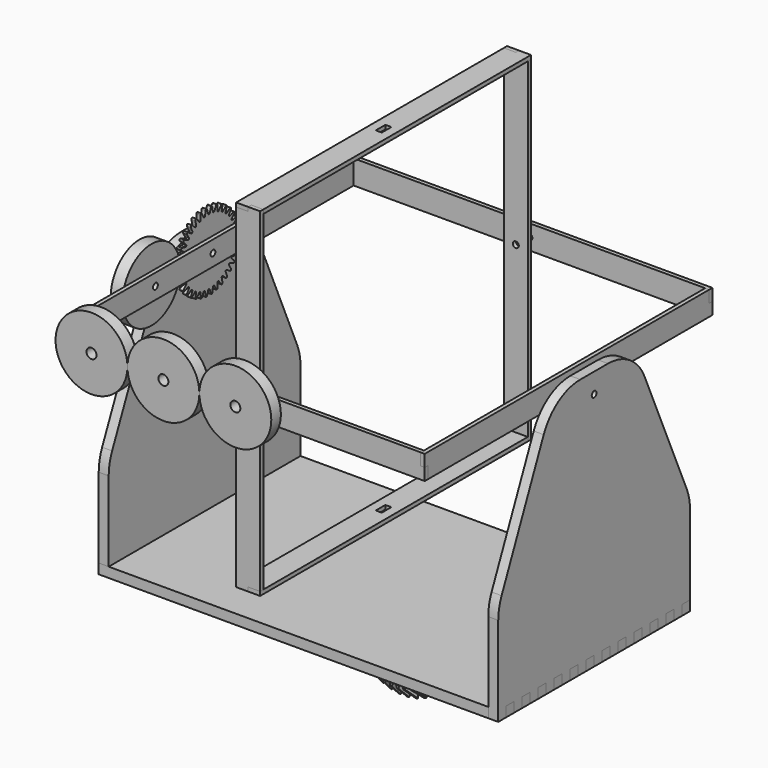
from build123d import *

# Parameters (mm, degrees)
F1_DEPTH  = 5
F2_R      = 1.5
F3_DEPTH  = 5
F4_R      = 1.5
F5_DEPTH  = 5
F6_R      = 1.5
F7_DEPTH  = 2
F8_R      = 1.5
F9_DEPTH  = 2
F10_R     = 1.5
F11_DEPTH = 2
F12_R     = 1.5
F13_DEPTH = 2
F14_R     = 1.5
F15_DEPTH = 2
F16_R     = 1.5
F17_DEPTH = 2
F18_W     = 3
F18_H     = 6
F19_DEPTH = 2
F20_R     = 1.5
F21_DEPTH = 2
F22_W     = 3
F22_H     = 6
F23_DEPTH = 2
F26_R     = 18
F26_R_2   = 2.5
F27_DEPTH = 6
F28_R     = 18
F28_R_2   = 2.5
F29_DEPTH = 6
F30_R     = 18
F30_R_2   = 2.5
F31_DEPTH = 6
F32_R     = 18
F32_R_2   = 2.5
F33_DEPTH = 6
F40_R     = 2.5
F41_DEPTH = 25


# Not quite as in the source:
# - a feature of the source that left no trace in its solid (it failed there, or was rolled back) is left out


with BuildPart() as f1:
    # F0 (on Top) → F1 (new body)
    with BuildSketch(Plane.XY):
        Polygon((100, 55), (100, 60), (-95, 60), (-95, 55), (-100, 55), (-100, 50), (-95, 50), (-95, 45), (-100, 45), (-100, 40), (-95, 40), (-95, 35), (-100, 35), (-100, 30), (-95, 30), (-95, 25), (-100, 25), (-100, 20), (-95, 20), (-95, 15), (-100, 15), (-100, 10), (-95, 10), (-95, 5), (-100, 5), (-100, 0), (-95, 0), (-95, -5), (-100, -5), (-100, -10), (-95, -10), (-95, -15), (-100, -15), (-100, -20), (-95, -20), (-95, -25), (-100, -25), (-100, -30), (-95, -30), (-95, -35), (-100, -35), (-100, -40), (-95, -40), (-95, -45), (-100, -45), (-100, -50), (-95, -50), (-95, -55), (-100, -55), (-100, -60), (95, -60), (95, -55), (100, -55), (100, -50), (95, -50), (95, -45), (100, -45), (100, -40), (95, -40), (95, -35), (100, -35), (100, -30), (95, -30), (95, -25), (100, -25), (100, -20), (95, -20), (95, -15), (100, -15), (100, -10), (95, -10), (95, -5), (100, -5), (100, 0), (95, 0), (95, 5), (100, 5), (100, 10), (95, 10), (95, 15), (100, 15), (100, 20), (95, 20), (95, 25), (100, 25), (100, 30), (95, 30), (95, 35), (100, 35), (100, 40), (95, 40), (95, 45), (100, 45), (100, 50), (95, 50), (95, 55), align=None)
    extrude(amount=F1_DEPTH)


with BuildPart() as f3:
    # F2 (on face) → F3 (new body)
    with BuildSketch(Plane.YZ.offset(100)):
        with BuildLine():
            Line((50, 0), (55, 0))
            Line((55, 0), (55, 5))
            Line((55, 5), (60, 5))
            Line((60, 5), (60, 44.7705385837))
            ThreePointArc((60, 44.7705385837), (59.4703732533, 49.8892134945), (57.9039333726, 54.7910094342))
            Line((57.9039333726, 54.7910094342), (31.5535440029, 115.0204708505))
            ThreePointArc((31.5535440029, 115.0204708505), (22.3333277558, 125.9226166057), (8.6496106304, 130))
            Line((8.6496106304, 130), (-8.6496106304, 130))
            ThreePointArc((-8.6496106304, 130), (-22.3333277558, 125.9226166057), (-31.5535440029, 115.0204708505))
            Line((-31.5535440029, 115.0204708505), (-57.9039333726, 54.7910094342))
            ThreePointArc((-57.9039333726, 54.7910094342), (-59.4703732533, 49.8892134945), (-60, 44.7705385837))
            Line((-60, 44.7705385837), (-60, 0))
            Line((-60, 0), (-55, 0))
            Line((-55, 0), (-55, 5))
            Line((-55, 5), (-50, 5))
            Line((-50, 5), (-50, 0))
            Line((-50, 0), (-45, 0))
            Line((-45, 0), (-45, 5))
            Line((-45, 5), (-40, 5))
            Line((-40, 5), (-40, 0))
            Line((-40, 0), (-35, 0))
            Line((-35, 0), (-35, 5))
            Line((-35, 5), (-30, 5))
            Line((-30, 5), (-30, 0))
            Line((-30, 0), (-25, 0))
            Line((-25, 0), (-25, 5))
            Line((-25, 5), (-20, 5))
            Line((-20, 5), (-20, 0))
            Line((-20, 0), (-15, 0))
            Line((-15, 0), (-15, 5))
            Line((-15, 5), (-10, 5))
            Line((-10, 5), (-10, 0))
            Line((-10, 0), (-5, 0))
            Line((-5, 0), (-5, 5))
            Line((-5, 5), (0, 5))
            Line((0, 5), (0, 0))
            Line((0, 0), (5, 0))
            Line((5, 0), (5, 5))
            Line((5, 5), (10, 5))
            Line((10, 5), (10, 0))
            Line((10, 0), (15, 0))
            Line((15, 0), (15, 5))
            Line((15, 5), (20, 5))
            Line((20, 5), (20, 0))
            Line((20, 0), (25, 0))
            Line((25, 0), (25, 5))
            Line((25, 5), (30, 5))
            Line((30, 5), (30, 0))
            Line((30, 0), (35, 0))
            Line((35, 0), (35, 5))
            Line((35, 5), (40, 5))
            Line((40, 5), (40, 0))
            Line((40, 0), (45, 0))
            Line((45, 0), (45, 5))
            Line((45, 5), (50, 5))
            Line((50, 5), (50, 0))
        make_face()
        with Locations((0, 120)):
            Circle(F2_R, mode=Mode.SUBTRACT)
    extrude(amount=-F3_DEPTH)


with BuildPart() as f5:
    # F4 (on face) → F5 (new body)
    with BuildSketch(Plane(origin=(-100, 0, 0), x_dir=(0, -1, 0), z_dir=(-1, 0, 0))):
        with BuildLine():
            Line((50, 0), (55, 0))
            Line((55, 0), (55, 5))
            Line((55, 5), (60, 5))
            Line((60, 5), (60, 45.0277700469))
            ThreePointArc((60, 45.0277700469), (59.4580269805, 50.2051164927), (57.8556067024, 55.1579843716))
            Line((57.8556067024, 55.1579843716), (31.2743152553, 115.1302143247))
            ThreePointArc((31.2743152553, 115.1302143247), (22.0522085049, 125.9553735128), (8.4187085529, 130))
            Line((8.4187085529, 130), (-8.9065918714, 130))
            ThreePointArc((-8.9065918714, 130), (-22.6250646146, 125.8998446308), (-31.8437077839, 114.9442804474))
            Line((-31.8437077839, 114.9442804474), (-57.9371159125, 54.7581734726))
            ThreePointArc((-57.9371159125, 54.7581734726), (-59.4788469685, 49.8918897851), (-60, 44.8138930252))
            Line((-60, 44.8138930252), (-60, 0))
            Line((-60, 0), (-55, 0))
            Line((-55, 0), (-55, 5))
            Line((-55, 5), (-50, 5))
            Line((-50, 5), (-50, 0))
            Line((-50, 0), (-45, 0))
            Line((-45, 0), (-45, 5))
            Line((-45, 5), (-40, 5))
            Line((-40, 5), (-40, 0))
            Line((-40, 0), (-35, 0))
            Line((-35, 0), (-35, 5))
            Line((-35, 5), (-30, 5))
            Line((-30, 5), (-30, 0))
            Line((-30, 0), (-25, 0))
            Line((-25, 0), (-25, 5))
            Line((-25, 5), (-20, 5))
            Line((-20, 5), (-20, 0))
            Line((-20, 0), (-15, 0))
            Line((-15, 0), (-15, 5))
            Line((-15, 5), (-10, 5))
            Line((-10, 5), (-10, 0))
            Line((-10, 0), (-5, 0))
            Line((-5, 0), (-5, 5))
            Line((-5, 5), (0, 5))
            Line((0, 5), (0, 0))
            Line((0, 0), (5, 0))
            Line((5, 0), (5, 5))
            Line((5, 5), (10, 5))
            Line((10, 5), (10, 0))
            Line((10, 0), (15, 0))
            Line((15, 0), (15, 5))
            Line((15, 5), (20, 5))
            Line((20, 5), (20, 0))
            Line((20, 0), (25, 0))
            Line((25, 0), (25, 5))
            Line((25, 5), (30, 5))
            Line((30, 5), (30, 0))
            Line((30, 0), (35, 0))
            Line((35, 0), (35, 5))
            Line((35, 5), (40, 5))
            Line((40, 5), (40, 0))
            Line((40, 0), (45, 0))
            Line((45, 0), (45, 5))
            Line((45, 5), (50, 5))
            Line((50, 5), (50, 0))
        make_face()
        with Locations((-0.2439416593, 120)):
            Circle(F4_R, mode=Mode.SUBTRACT)
    extrude(amount=-F5_DEPTH)


with BuildPart() as f7:
    # F6 (on face) → F7 (new body)
    with BuildSketch(Plane.YZ.offset(-95)):
        with BuildLine():
            ThreePointArc((-0.9074454432, 138.9766193212), (-1.1059043827, 139.2442584986), (-1.4284580066, 139.3277799904))
            ThreePointArc((-1.4284580066, 139.3277799904), (-1.44687975, 139.326177143), (-1.4652999573, 139.3245567374))
            ThreePointArc((-1.4652999573, 139.3245567374), (-1.7684499121, 139.1862932757), (-1.9174187589, 138.8882581056))
            Line((-1.9174187589, 138.8882581056), (-2.2042135214, 136.5840744477))
            ThreePointArc((-2.2042135214, 136.5840744477), (-2.3348708966, 136.3046577179), (-2.6046356928, 136.1550849487))
            ThreePointArc((-2.6046356928, 136.1550849487), (-2.9092885812, 136.2033723819), (-3.1276325025, 136.4212507668))
            Line((-3.1276325025, 136.4212507668), (-4.1852086494, 138.4883855613))
            ThreePointArc((-4.1852086494, 138.4883855613), (-4.427127607, 138.7174966651), (-4.7592842715, 138.7437384288))
            ThreePointArc((-4.7592842715, 138.7437384288), (-4.7771478157, 138.73896103), (-4.7950067982, 138.7341666066))
            ThreePointArc((-4.7950067982, 138.7341666066), (-5.0695420259, 138.5453622404), (-5.164494437, 138.2259867254))
            Line((-5.164494437, 138.2259867254), (-5.0468148493, 135.9070074068))
            ThreePointArc((-5.0468148493, 135.9070074068), (-5.1269670395, 135.6091472299), (-5.3666604635, 135.415002642))
            ThreePointArc((-5.3666604635, 135.415002642), (-5.6750700147, 135.4096540616), (-5.9279309858, 135.5863073602))
            Line((-5.9279309858, 135.5863073602), (-7.3283943647, 137.4383915618))
            ThreePointArc((-7.3283943647, 137.4383915618), (-7.6064227554, 137.6220131669), (-7.9380900483, 137.5901778597))
            ThreePointArc((-7.9380900483, 137.5901778597), (-7.9548526185, 137.5823710685), (-7.97160774, 137.5745483034))
            ThreePointArc((-7.97160774, 137.5745483034), (-8.2091866266, 137.3409397577), (-8.247237521, 137.0099279613))
            Line((-8.247237521, 137.0099279613), (-7.728659218, 134.7466139953))
            ThreePointArc((-7.728659218, 134.7466139953), (-7.7558708394, 134.439360702), (-7.9582099279, 134.2065432803))
            ThreePointArc((-7.9582099279, 134.2065432803), (-8.2610052737, 134.1477212004), (-8.5407002418, 134.2777818916))
            Line((-8.5407002418, 134.2777818916), (-10.2414984817, 135.8585408589))
            ThreePointArc((-10.2414984817, 135.8585408589), (-10.5471885535, 135.9910937158), (-10.8682889319, 135.9021486375))
            ThreePointArc((-10.8682889319, 135.9021486375), (-10.883441206, 135.8915496592), (-10.8985833706, 135.8809362432))
            ThreePointArc((-10.8985833706, 135.8809362432), (-11.0919872018, 135.6096215955), (-11.0719804224, 135.2770311436))
            Line((-11.0719804224, 135.2770311436), (-10.1682601434, 133.1381521796))
            ThreePointArc((-10.1682601434, 133.1381521796), (-10.1417043847, 132.8308415058), (-10.3005411667, 132.5664252899))
            ThreePointArc((-10.3005411667, 132.5664252899), (-10.5885220239, 132.4559169895), (-10.886552599, 132.5354332451))
            Line((-10.886552599, 132.5354332451), (-12.8360078059, 133.7968364168))
            ThreePointArc((-12.8360078059, 133.7968364168), (-13.1600713207, 133.8742929741), (-13.4608483121, 133.7309406758))
            ThreePointArc((-13.4608483121, 133.7309406758), (-13.4739298958, 133.717871555), (-13.4869990165, 133.7047899713))
            ThreePointArc((-13.4869990165, 133.7047899713), (-13.6303513148, 133.40401298), (-13.5528947575, 133.0799494651))
            Line((-13.5528947575, 133.0799494651), (-12.2914915858, 131.1304942582))
            ThreePointArc((-12.2914915858, 131.1304942582), (-12.2119753303, 130.8324636832), (-12.3224836306, 130.5444828259))
            ThreePointArc((-12.3224836306, 130.5444828259), (-12.5868998465, 130.3856460439), (-12.8942105204, 130.4122018027))
            Line((-12.8942105204, 130.4122018027), (-15.0330894843, 131.3159220817))
            ThreePointArc((-15.0330894843, 131.3159220817), (-15.3656799363, 131.335928861), (-15.6369945839, 131.1425250298))
            ThreePointArc((-15.6369945839, 131.1425250298), (-15.647608, 131.1273828652), (-15.6582069782, 131.1122305911))
            ThreePointArc((-15.6582069782, 131.1122305911), (-15.7471520566, 130.7911302128), (-15.6145991996, 130.4854401409))
            Line((-15.6145991996, 130.4854401409), (-14.0338402323, 128.7846419011))
            ThreePointArc((-14.0338402323, 128.7846419011), (-13.9037795411, 128.504946933), (-13.962601621, 128.2021515871))
            ThreePointArc((-13.962601621, 128.2021515871), (-14.1954190427, 127.9998124987), (-14.502672336, 127.9726008773))
            Line((-14.502672336, 127.9726008773), (-16.7659863021, 128.4911791803))
            ThreePointArc((-16.7659863021, 128.4911791803), (-17.0969980985, 128.4531282858), (-17.3306066441, 128.2155493993))
            ThreePointArc((-17.3306066441, 128.2155493993), (-17.3384294093, 128.1987942778), (-17.3462362005, 128.1820317075))
            ThreePointArc((-17.3462362005, 128.1820317075), (-17.3780715077, 127.8503644147), (-17.1944499025, 127.5723360239))
            Line((-17.1944499025, 127.5723360239), (-15.342365701, 126.171872645))
            ThreePointArc((-15.342365701, 126.171872645), (-15.1657124024, 125.919011674), (-15.1710609827, 125.6106021228))
            ThreePointArc((-15.1710609827, 125.6106021228), (-15.3652055707, 125.3709086988), (-15.6630657476, 125.2907565086))
            Line((-15.6630657476, 125.2907565086), (-17.9820450661, 125.4084360962))
            ThreePointArc((-17.9820450661, 125.4084360962), (-18.3014205811, 125.3134836851), (-18.4902249473, 125.0389484574))
            ThreePointArc((-18.4902249473, 125.0389484574), (-18.4950193708, 125.021089475), (-18.4997967695, 125.0032259308))
            ThreePointArc((-18.4997967695, 125.0032259308), (-18.4735550058, 124.6710692663), (-18.2444439021, 124.4291503086))
            Line((-18.2444439021, 124.4291503086), (-16.1773091075, 123.3715741617))
            ThreePointArc((-16.1773091075, 123.3715741617), (-15.9594307227, 123.1532302404), (-15.9111432895, 122.8485773521))
            ThreePointArc((-15.9111432895, 122.8485773521), (-16.0607160587, 122.5788125559), (-16.3401327884, 122.4481551806))
            Line((-16.3401327884, 122.4481551806), (-18.6443164463, 122.1613604182))
            ThreePointArc((-18.6443164463, 122.1613604182), (-18.9423516165, 122.0123915714), (-19.0806150781, 121.7092416166))
            ThreePointArc((-19.0806150781, 121.7092416166), (-19.0822354837, 121.6908214093), (-19.0838383312, 121.6723996659))
            ThreePointArc((-19.0838383312, 121.6723996659), (-19.0003168394, 121.3498460419), (-18.7326776619, 121.1513871025))
            Line((-18.7326776619, 121.1513871025), (-16.5133011191, 120.4688321037))
            ThreePointArc((-16.5133011191, 120.4688321037), (-16.2608177724, 120.2916395016), (-16.160361515, 120))
            ThreePointArc((-16.160361515, 120), (-16.2608177724, 119.7083604984), (-16.5133011191, 119.5311678963))
            Line((-16.5133011191, 119.5311678963), (-18.7326776619, 118.8486128975))
            ThreePointArc((-18.7326776619, 118.8486128975), (-19.0003168394, 118.6501539581), (-19.0838383312, 118.3276003341))
            ThreePointArc((-19.0838383312, 118.3276003341), (-19.0822354837, 118.3091785907), (-19.0806150781, 118.2907583834))
            ThreePointArc((-19.0806150781, 118.2907583834), (-18.9423516165, 117.9876084286), (-18.6443164463, 117.8386395818))
            Line((-18.6443164463, 117.8386395818), (-16.3401327884, 117.5518448194))
            ThreePointArc((-16.3401327884, 117.5518448194), (-16.0607160587, 117.4211874442), (-15.9111432895, 117.1514226479))
            ThreePointArc((-15.9111432895, 117.1514226479), (-15.9594307227, 116.8467697596), (-16.1773091075, 116.6284258383))
            Line((-16.1773091075, 116.6284258383), (-18.2444439021, 115.5708496914))
            ThreePointArc((-18.2444439021, 115.5708496914), (-18.4735550058, 115.3289307337), (-18.4997967695, 114.9967740692))
            ThreePointArc((-18.4997967695, 114.9967740692), (-18.4950193708, 114.978910525), (-18.4902249473, 114.9610515426))
            ThreePointArc((-18.4902249473, 114.9610515426), (-18.3014205811, 114.6865163149), (-17.9820450661, 114.5915639038))
            Line((-17.9820450661, 114.5915639038), (-15.6630657476, 114.7092434914))
            ThreePointArc((-15.6630657476, 114.7092434914), (-15.3652055707, 114.6290913012), (-15.1710609827, 114.3893978772))
            ThreePointArc((-15.1710609827, 114.3893978772), (-15.1657124024, 114.080988326), (-15.342365701, 113.828127355))
            Line((-15.342365701, 113.828127355), (-17.1944499025, 112.4276639761))
            ThreePointArc((-17.1944499025, 112.4276639761), (-17.3780715077, 112.1496355853), (-17.3462362005, 111.8179682925))
            ThreePointArc((-17.3462362005, 111.8179682925), (-17.3384294093, 111.8012057222), (-17.3306066441, 111.7844506007))
            ThreePointArc((-17.3306066441, 111.7844506007), (-17.0969980985, 111.5468717142), (-16.7659863021, 111.5088208197))
            Line((-16.7659863021, 111.5088208197), (-14.502672336, 112.0273991227))
            ThreePointArc((-14.502672336, 112.0273991227), (-14.1954190427, 112.0001875013), (-13.962601621, 111.7978484129))
            ThreePointArc((-13.962601621, 111.7978484129), (-13.9037795411, 111.495053067), (-14.0338402323, 111.2153580989))
            Line((-14.0338402323, 111.2153580989), (-15.6145991996, 109.5145598591))
            ThreePointArc((-15.6145991996, 109.5145598591), (-15.7471520566, 109.2088697872), (-15.6582069782, 108.8877694089))
            ThreePointArc((-15.6582069782, 108.8877694089), (-15.647608, 108.8726171348), (-15.6369945839, 108.8574749702))
            ThreePointArc((-15.6369945839, 108.8574749702), (-15.3656799363, 108.664071139), (-15.0330894843, 108.6840779183))
            Line((-15.0330894843, 108.6840779183), (-12.8942105204, 109.5877981973))
            ThreePointArc((-12.8942105204, 109.5877981973), (-12.5868998465, 109.6143539561), (-12.3224836306, 109.4555171741))
            ThreePointArc((-12.3224836306, 109.4555171741), (-12.2119753303, 109.1675363168), (-12.2914915858, 108.8695057418))
            Line((-12.2914915858, 108.8695057418), (-13.5528947575, 106.9200505349))
            ThreePointArc((-13.5528947575, 106.9200505349), (-13.6303513148, 106.59598702), (-13.4869990165, 106.2952100287))
            ThreePointArc((-13.4869990165, 106.2952100287), (-13.4739298958, 106.282128445), (-13.4608483121, 106.2690593242))
            ThreePointArc((-13.4608483121, 106.2690593242), (-13.1600713207, 106.1257070259), (-12.8360078059, 106.2031635832))
            Line((-12.8360078059, 106.2031635832), (-10.886552599, 107.4645667549))
            ThreePointArc((-10.886552599, 107.4645667549), (-10.5885220239, 107.5440830105), (-10.3005411667, 107.4335747102))
            ThreePointArc((-10.3005411667, 107.4335747102), (-10.1417043847, 107.1691584942), (-10.1682601434, 106.8618478204))
            Line((-10.1682601434, 106.8618478204), (-11.0719804224, 104.7229688564))
            ThreePointArc((-11.0719804224, 104.7229688564), (-11.0919872018, 104.3903784045), (-10.8985833706, 104.1190637568))
            ThreePointArc((-10.8985833706, 104.1190637568), (-10.883441206, 104.1084503408), (-10.8682889319, 104.0978513625))
            ThreePointArc((-10.8682889319, 104.0978513625), (-10.5471885535, 104.0089062842), (-10.2414984817, 104.1414591411))
            Line((-10.2414984817, 104.1414591411), (-8.5407002418, 105.7222181084))
            ThreePointArc((-8.5407002418, 105.7222181084), (-8.2610052737, 105.8522787996), (-7.9582099279, 105.7934567197))
            ThreePointArc((-7.9582099279, 105.7934567197), (-7.7558708394, 105.560639298), (-7.728659218, 105.2533860047))
            Line((-7.728659218, 105.2533860047), (-8.247237521, 102.9900720387))
            ThreePointArc((-8.247237521, 102.9900720387), (-8.2091866266, 102.6590602423), (-7.97160774, 102.4254516966))
            ThreePointArc((-7.97160774, 102.4254516966), (-7.9548526185, 102.4176289315), (-7.9380900483, 102.4098221403))
            ThreePointArc((-7.9380900483, 102.4098221403), (-7.6064227554, 102.3779868331), (-7.3283943647, 102.5616084382))
            Line((-7.3283943647, 102.5616084382), (-5.9279309858, 104.4136926398))
            ThreePointArc((-5.9279309858, 104.4136926398), (-5.6750700147, 104.5903459384), (-5.3666604636, 104.5849973581))
            ThreePointArc((-5.3666604636, 104.5849973581), (-5.1269670395, 104.3908527701), (-5.0468148493, 104.0929925932))
            Line((-5.0468148493, 104.0929925932), (-5.164494437, 101.7740132746))
            ThreePointArc((-5.164494437, 101.7740132746), (-5.0695420259, 101.4546377596), (-4.7950067982, 101.2658333934))
            ThreePointArc((-4.7950067982, 101.2658333934), (-4.7771478157, 101.26103897), (-4.7592842715, 101.2562615712))
            ThreePointArc((-4.7592842715, 101.2562615712), (-4.427127607, 101.2825033349), (-4.1852086494, 101.5116144387))
            Line((-4.1852086494, 101.5116144387), (-3.1276325025, 103.5787492332))
            ThreePointArc((-3.1276325025, 103.5787492332), (-2.9092885812, 103.7966276181), (-2.6046356928, 103.8449150513))
            ThreePointArc((-2.6046356928, 103.8449150513), (-2.3348708966, 103.6953422821), (-2.2042135214, 103.4159255523))
            Line((-2.2042135214, 103.4159255523), (-1.9174187589, 101.1117418944))
            ThreePointArc((-1.9174187589, 101.1117418944), (-1.7684499121, 100.8137067243), (-1.4652999573, 100.6754432626))
            ThreePointArc((-1.4652999573, 100.6754432626), (-1.44687975, 100.673822857), (-1.4284580066, 100.6722200096))
            ThreePointArc((-1.4284580066, 100.6722200096), (-1.1059043827, 100.7557415014), (-0.9074454432, 101.0233806788))
            Line((-0.9074454432, 101.0233806788), (-0.2248904444, 103.2427572216))
            ThreePointArc((-0.2248904444, 103.2427572216), (-0.0476978424, 103.4952405683), (0.2439416592, 103.5956968258))
            ThreePointArc((0.2439416592, 103.5956968258), (0.5355811609, 103.4952405683), (0.7127737629, 103.2427572216))
            Line((0.7127737629, 103.2427572216), (1.3953287617, 101.0233806788))
            ThreePointArc((1.3953287617, 101.0233806788), (1.5937877012, 100.7557415014), (1.9163413251, 100.6722200096))
            ThreePointArc((1.9163413251, 100.6722200096), (1.9347630686, 100.673822857), (1.9531832758, 100.6754432626))
            ThreePointArc((1.9531832758, 100.6754432626), (2.2563332306, 100.8137067243), (2.4053020774, 101.1117418944))
            Line((2.4053020774, 101.1117418944), (2.6920968399, 103.4159255523))
            ThreePointArc((2.6920968399, 103.4159255523), (2.8227542151, 103.6953422821), (3.0925190113, 103.8449150513))
            ThreePointArc((3.0925190113, 103.8449150513), (3.3971718997, 103.7966276181), (3.615515821, 103.5787492332))
            Line((3.615515821, 103.5787492332), (4.6730919679, 101.5116144387))
            ThreePointArc((4.6730919679, 101.5116144387), (4.9150109255, 101.2825033349), (5.24716759, 101.2562615712))
            ThreePointArc((5.24716759, 101.2562615712), (5.2650311342, 101.26103897), (5.2828901167, 101.2658333934))
            ThreePointArc((5.2828901167, 101.2658333934), (5.5574253444, 101.4546377596), (5.6523777555, 101.7740132746))
            Line((5.6523777555, 101.7740132746), (5.5346981678, 104.0929925932))
            ThreePointArc((5.5346981678, 104.0929925932), (5.614850358, 104.3908527701), (5.8545437821, 104.584997358))
            ThreePointArc((5.8545437821, 104.584997358), (6.1629533332, 104.5903459384), (6.4158143043, 104.4136926398))
            Line((6.4158143043, 104.4136926398), (7.8162776832, 102.5616084382))
            ThreePointArc((7.8162776832, 102.5616084382), (8.0943060739, 102.3779868331), (8.4259733668, 102.4098221403))
            ThreePointArc((8.4259733668, 102.4098221403), (8.442735937, 102.4176289315), (8.4594910585, 102.4254516966))
            ThreePointArc((8.4594910585, 102.4254516966), (8.6970699451, 102.6590602423), (8.7351208395, 102.9900720387))
            Line((8.7351208395, 102.9900720387), (8.2165425365, 105.2533860047))
            ThreePointArc((8.2165425365, 105.2533860047), (8.2437541579, 105.560639298), (8.4460932464, 105.7934567197))
            ThreePointArc((8.4460932464, 105.7934567197), (8.7488885922, 105.8522787996), (9.0285835603, 105.7222181084))
            Line((9.0285835603, 105.7222181084), (10.7293818002, 104.1414591411))
            ThreePointArc((10.7293818002, 104.1414591411), (11.0350718721, 104.0089062842), (11.3561722504, 104.0978513625))
            ThreePointArc((11.3561722504, 104.0978513625), (11.3713245245, 104.1084503408), (11.3864666891, 104.1190637568))
            ThreePointArc((11.3864666891, 104.1190637568), (11.5798705203, 104.3903784045), (11.5598637409, 104.7229688564))
            Line((11.5598637409, 104.7229688564), (10.6561434619, 106.8618478204))
            ThreePointArc((10.6561434619, 106.8618478204), (10.6295877032, 107.1691584942), (10.7884244852, 107.4335747101))
            ThreePointArc((10.7884244852, 107.4335747101), (11.0764053424, 107.5440830105), (11.3744359175, 107.4645667549))
            Line((11.3744359175, 107.4645667549), (13.3238911244, 106.2031635832))
            ThreePointArc((13.3238911244, 106.2031635832), (13.6479546392, 106.1257070259), (13.9487316306, 106.2690593242))
            ThreePointArc((13.9487316306, 106.2690593242), (13.9618132143, 106.282128445), (13.9748823351, 106.2952100287))
            ThreePointArc((13.9748823351, 106.2952100287), (14.1182346333, 106.59598702), (14.040778076, 106.9200505349))
            Line((14.040778076, 106.9200505349), (12.7793749043, 108.8695057418))
            ThreePointArc((12.7793749043, 108.8695057418), (12.6998586488, 109.1675363168), (12.8103669491, 109.4555171741))
            ThreePointArc((12.8103669491, 109.4555171741), (13.074783165, 109.6143539561), (13.3820938389, 109.5877981973))
            Line((13.3820938389, 109.5877981973), (15.5209728028, 108.6840779183))
            ThreePointArc((15.5209728028, 108.6840779183), (15.8535632548, 108.664071139), (16.1248779024, 108.8574749702))
            ThreePointArc((16.1248779024, 108.8574749702), (16.1354913185, 108.8726171348), (16.1460902968, 108.8877694089))
            ThreePointArc((16.1460902968, 108.8877694089), (16.2350353751, 109.2088697872), (16.1024825181, 109.5145598591))
            Line((16.1024825181, 109.5145598591), (14.5217235509, 111.2153580989))
            ThreePointArc((14.5217235509, 111.2153580989), (14.3916628596, 111.495053067), (14.4504849395, 111.7978484129))
            ThreePointArc((14.4504849395, 111.7978484129), (14.6833023613, 112.0001875013), (14.9905556545, 112.0273991227))
            Line((14.9905556545, 112.0273991227), (17.2538696206, 111.5088208197))
            ThreePointArc((17.2538696206, 111.5088208197), (17.584881417, 111.5468717142), (17.8184899626, 111.7844506007))
            ThreePointArc((17.8184899626, 111.7844506007), (17.8263127278, 111.8012057222), (17.834119519, 111.8179682925))
            ThreePointArc((17.834119519, 111.8179682925), (17.8659548262, 112.1496355853), (17.682333221, 112.4276639761))
            Line((17.682333221, 112.4276639761), (15.8302490195, 113.828127355))
            ThreePointArc((15.8302490195, 113.828127355), (15.6535957209, 114.080988326), (15.6589443012, 114.3893978772))
            ThreePointArc((15.6589443012, 114.3893978772), (15.8530888892, 114.6290913012), (16.1509490661, 114.7092434914))
            Line((16.1509490661, 114.7092434914), (18.4699283846, 114.5915639038))
            ThreePointArc((18.4699283846, 114.5915639038), (18.7893038996, 114.6865163149), (18.9781082658, 114.9610515426))
            ThreePointArc((18.9781082658, 114.9610515426), (18.9829026893, 114.978910525), (18.987680088, 114.9967740692))
            ThreePointArc((18.987680088, 114.9967740692), (18.9614383244, 115.3289307337), (18.7323272206, 115.5708496914))
            Line((18.7323272206, 115.5708496914), (16.6651924261, 116.6284258383))
            ThreePointArc((16.6651924261, 116.6284258383), (16.4473140412, 116.8467697596), (16.399026608, 117.1514226479))
            ThreePointArc((16.399026608, 117.1514226479), (16.5485993772, 117.4211874441), (16.8280161069, 117.5518448194))
            Line((16.8280161069, 117.5518448194), (19.1321997648, 117.8386395818))
            ThreePointArc((19.1321997648, 117.8386395818), (19.430234935, 117.9876084286), (19.5684983966, 118.2907583834))
            ThreePointArc((19.5684983966, 118.2907583834), (19.5701188022, 118.3091785907), (19.5717216497, 118.3276003341))
            ThreePointArc((19.5717216497, 118.3276003341), (19.4882001579, 118.6501539581), (19.2205609804, 118.8486128975))
            Line((19.2205609804, 118.8486128975), (17.0011844376, 119.5311678963))
            ThreePointArc((17.0011844376, 119.5311678963), (16.7487010909, 119.7083604984), (16.6482448335, 120))
            ThreePointArc((16.6482448335, 120), (16.7487010909, 120.2916395016), (17.0011844376, 120.4688321037))
            Line((17.0011844376, 120.4688321037), (19.2205609804, 121.1513871025))
            ThreePointArc((19.2205609804, 121.1513871025), (19.4882001579, 121.3498460419), (19.5717216497, 121.6723996659))
            ThreePointArc((19.5717216497, 121.6723996659), (19.5701188022, 121.6908214093), (19.5684983966, 121.7092416166))
            ThreePointArc((19.5684983966, 121.7092416166), (19.430234935, 122.0123915714), (19.1321997648, 122.1613604182))
            Line((19.1321997648, 122.1613604182), (16.8280161069, 122.4481551806))
            ThreePointArc((16.8280161069, 122.4481551806), (16.5485993772, 122.5788125558), (16.399026608, 122.8485773521))
            ThreePointArc((16.399026608, 122.8485773521), (16.4473140412, 123.1532302404), (16.6651924261, 123.3715741617))
            Line((16.6651924261, 123.3715741617), (18.7323272206, 124.4291503086))
            ThreePointArc((18.7323272206, 124.4291503086), (18.9614383244, 124.6710692663), (18.987680088, 125.0032259308))
            ThreePointArc((18.987680088, 125.0032259308), (18.9829026893, 125.021089475), (18.9781082658, 125.0389484574))
            ThreePointArc((18.9781082658, 125.0389484574), (18.7893038996, 125.3134836851), (18.4699283846, 125.4084360962))
            Line((18.4699283846, 125.4084360962), (16.1509490661, 125.2907565086))
            ThreePointArc((16.1509490661, 125.2907565086), (15.8530888892, 125.3709086988), (15.6589443012, 125.6106021228))
            ThreePointArc((15.6589443012, 125.6106021228), (15.6535957209, 125.919011674), (15.8302490195, 126.171872645))
            Line((15.8302490195, 126.171872645), (17.682333221, 127.5723360239))
            ThreePointArc((17.682333221, 127.5723360239), (17.8659548262, 127.8503644147), (17.834119519, 128.1820317075))
            ThreePointArc((17.834119519, 128.1820317075), (17.8263127278, 128.1987942778), (17.8184899626, 128.2155493993))
            ThreePointArc((17.8184899626, 128.2155493993), (17.584881417, 128.4531282858), (17.2538696206, 128.4911791803))
            Line((17.2538696206, 128.4911791803), (14.9905556545, 127.9726008773))
            ThreePointArc((14.9905556545, 127.9726008773), (14.6833023613, 127.9998124987), (14.4504849395, 128.2021515871))
            ThreePointArc((14.4504849395, 128.2021515871), (14.3916628596, 128.504946933), (14.5217235509, 128.7846419011))
            Line((14.5217235509, 128.7846419011), (16.1024825181, 130.4854401409))
            ThreePointArc((16.1024825181, 130.4854401409), (16.2350353751, 130.7911302128), (16.1460902968, 131.1122305911))
            ThreePointArc((16.1460902968, 131.1122305911), (16.1354913185, 131.1273828652), (16.1248779024, 131.1425250298))
            ThreePointArc((16.1248779024, 131.1425250298), (15.8535632548, 131.335928861), (15.5209728028, 131.3159220817))
            Line((15.5209728028, 131.3159220817), (13.3820938389, 130.4122018027))
            ThreePointArc((13.3820938389, 130.4122018027), (13.0747831651, 130.3856460439), (12.8103669491, 130.5444828259))
            ThreePointArc((12.8103669491, 130.5444828259), (12.6998586488, 130.8324636832), (12.7793749043, 131.1304942582))
            Line((12.7793749043, 131.1304942582), (14.040778076, 133.0799494651))
            ThreePointArc((14.040778076, 133.0799494651), (14.1182346333, 133.40401298), (13.9748823351, 133.7047899713))
            ThreePointArc((13.9748823351, 133.7047899713), (13.9618132143, 133.717871555), (13.9487316306, 133.7309406758))
            ThreePointArc((13.9487316306, 133.7309406758), (13.6479546392, 133.8742929741), (13.3238911244, 133.7968364168))
            Line((13.3238911244, 133.7968364168), (11.3744359175, 132.5354332451))
            ThreePointArc((11.3744359175, 132.5354332451), (11.0764053424, 132.4559169895), (10.7884244852, 132.5664252898))
            ThreePointArc((10.7884244852, 132.5664252898), (10.6295877032, 132.8308415058), (10.6561434619, 133.1381521796))
            Line((10.6561434619, 133.1381521796), (11.5598637409, 135.2770311436))
            ThreePointArc((11.5598637409, 135.2770311436), (11.5798705203, 135.6096215955), (11.3864666891, 135.8809362432))
            ThreePointArc((11.3864666891, 135.8809362432), (11.3713245245, 135.8915496592), (11.3561722504, 135.9021486375))
            ThreePointArc((11.3561722504, 135.9021486375), (11.0350718721, 135.9910937158), (10.7293818002, 135.8585408589))
            Line((10.7293818002, 135.8585408589), (9.0285835603, 134.2777818916))
            ThreePointArc((9.0285835603, 134.2777818916), (8.7488885923, 134.1477212004), (8.4460932464, 134.2065432803))
            ThreePointArc((8.4460932464, 134.2065432803), (8.2437541579, 134.439360702), (8.2165425365, 134.7466139953))
            Line((8.2165425365, 134.7466139953), (8.7351208395, 137.0099279613))
            ThreePointArc((8.7351208395, 137.0099279613), (8.6970699451, 137.3409397577), (8.4594910585, 137.5745483034))
            ThreePointArc((8.4594910585, 137.5745483034), (8.442735937, 137.5823710685), (8.4259733668, 137.5901778597))
            ThreePointArc((8.4259733668, 137.5901778597), (8.0943060739, 137.6220131669), (7.8162776832, 137.4383915618))
            Line((7.8162776832, 137.4383915618), (6.4158143043, 135.5863073602))
            ThreePointArc((6.4158143043, 135.5863073602), (6.1629533332, 135.4096540616), (5.8545437821, 135.4150026419))
            ThreePointArc((5.8545437821, 135.4150026419), (5.614850358, 135.6091472299), (5.5346981678, 135.9070074068))
            Line((5.5346981678, 135.9070074068), (5.6523777555, 138.2259867254))
            ThreePointArc((5.6523777555, 138.2259867254), (5.5574253444, 138.5453622404), (5.2828901167, 138.7341666066))
            ThreePointArc((5.2828901167, 138.7341666066), (5.2650311342, 138.73896103), (5.24716759, 138.7437384288))
            ThreePointArc((5.24716759, 138.7437384288), (4.9150109255, 138.7174966651), (4.6730919679, 138.4883855613))
            Line((4.6730919679, 138.4883855613), (3.615515821, 136.4212507668))
            ThreePointArc((3.615515821, 136.4212507668), (3.3971718997, 136.2033723819), (3.0925190114, 136.1550849487))
            ThreePointArc((3.0925190114, 136.1550849487), (2.8227542151, 136.3046577179), (2.6920968399, 136.5840744477))
            Line((2.6920968399, 136.5840744477), (2.4053020774, 138.8882581056))
            ThreePointArc((2.4053020774, 138.8882581056), (2.2563332306, 139.1862932757), (1.9531832758, 139.3245567374))
            ThreePointArc((1.9531832758, 139.3245567374), (1.9347630686, 139.326177143), (1.9163413251, 139.3277799904))
            ThreePointArc((1.9163413251, 139.3277799904), (1.5937877012, 139.2442584986), (1.3953287617, 138.9766193212))
            Line((1.3953287617, 138.9766193212), (0.7127737629, 136.7572427784))
            ThreePointArc((0.7127737629, 136.7572427784), (0.5355811609, 136.5047594317), (0.2439416593, 136.4043031742))
            ThreePointArc((0.2439416593, 136.4043031742), (-0.0476978424, 136.5047594317), (-0.2248904444, 136.7572427784))
            Line((-0.2248904444, 136.7572427784), (-0.9074454432, 138.9766193212))
        make_face()
        with BuildLine():
            ThreePointArc((-10.2852554216, 107.4207006941), (-10.2928339664, 107.4272140806), (-10.3005411667, 107.4335747102))
            ThreePointArc((-10.3005411667, 107.4335747102), (-10.3081435053, 107.440060309), (-10.3158739393, 107.446392681))
            Line((-10.3158739393, 107.446392681), (-10.3002843799, 107.4338807368))
            Line((-10.3002843799, 107.4338807368), (-10.2852554216, 107.4207006941))
        make_face(mode=Mode.SUBTRACT)
        with BuildLine():
            ThreePointArc((-12.3096656598, 109.4401844015), (-12.3159980317, 109.4479148355), (-12.3224836306, 109.4555171741))
            ThreePointArc((-12.3224836306, 109.4555171741), (-12.3288442602, 109.4632243744), (-12.3353576467, 109.4708029192))
            Line((-12.3353576467, 109.4708029192), (-12.322177604, 109.4557739609))
            Line((-12.322177604, 109.4557739609), (-12.3096656598, 109.4401844015))
        make_face(mode=Mode.SUBTRACT)
        with BuildLine():
            ThreePointArc((-5.3478933889, 104.5781277729), (-5.3572426009, 104.5816563391), (-5.3666604636, 104.5849973581))
            ThreePointArc((-5.3666604636, 104.5849973581), (-5.3760225305, 104.5884916745), (-5.3854525611, 104.5917981936))
            Line((-5.3854525611, 104.5917981936), (-5.3665238301, 104.5853727553))
            Line((-5.3665238301, 104.5853727553), (-5.3478933889, 104.5781277729))
        make_face(mode=Mode.SUBTRACT)
        with BuildLine():
            ThreePointArc((-2.5849608413, 103.8414086988), (-2.5947807468, 103.8432601846), (-2.6046356928, 103.8449150513))
            ThreePointArc((-2.6046356928, 103.8449150513), (-2.6144623106, 103.8467305753), (-2.6243232489, 103.8483493533))
            Line((-2.6243232489, 103.8483493533), (-2.6045663222, 103.8453084715))
            Line((-2.6045663222, 103.8453084715), (-2.5849608413, 103.8414086988))
        make_face(mode=Mode.SUBTRACT)
        with BuildLine():
            ThreePointArc((-7.9409208582, 105.7834326307), (-7.9495153055, 105.7885310637), (-7.9582099279, 105.7934567197))
            ThreePointArc((-7.9582099279, 105.7934567197), (-7.9668229823, 105.7985236555), (-7.9755355785, 105.8034174488))
            Line((-7.9755355785, 105.8034174488), (-7.9580101832, 105.7938026877))
            Line((-7.9580101832, 105.7938026877), (-7.9409208582, 105.7834326307))
        make_face(mode=Mode.SUBTRACT)
        with BuildLine():
            ThreePointArc((-15.1642601472, 114.3706057797), (-15.1675666662, 114.3800358103), (-15.1710609827, 114.3893978772))
            ThreePointArc((-15.1710609827, 114.3893978772), (-15.1744020016, 114.3988157399), (-15.1779305679, 114.4081649519))
            Line((-15.1779305679, 114.4081649519), (-15.1706855855, 114.3895345106))
            Line((-15.1706855855, 114.3895345106), (-15.1642601472, 114.3706057797))
        make_face(mode=Mode.SUBTRACT)
        with BuildLine():
            ThreePointArc((-13.952640892, 111.7805227623), (-13.9575346852, 111.7892353585), (-13.962601621, 111.7978484129))
            ThreePointArc((-13.962601621, 111.7978484129), (-13.967527277, 111.8065430352), (-13.9726257101, 111.8151374826))
            Line((-13.9726257101, 111.8151374826), (-13.9622556531, 111.7980481576))
            Line((-13.9622556531, 111.7980481576), (-13.952640892, 111.7805227623))
        make_face(mode=Mode.SUBTRACT)
        with BuildLine():
            ThreePointArc((-15.9077089874, 117.1317350919), (-15.9093277654, 117.1415960301), (-15.9111432895, 117.1514226479))
            ThreePointArc((-15.9111432895, 117.1514226479), (-15.9127981561, 117.1612775939), (-15.9146496419, 117.1710974995))
            Line((-15.9146496419, 117.1710974995), (-15.9107498693, 117.1514920185))
            Line((-15.9107498693, 117.1514920185), (-15.9077089874, 117.1317350919))
        make_face(mode=Mode.SUBTRACT)
        with BuildLine():
            ThreePointArc((-16.1603980959, 119.9800151819), (-16.160279947, 119.9900074082), (-16.160361515, 120))
            ThreePointArc((-16.160361515, 120), (-16.160279947, 120.0099925918), (-16.1603980959, 120.0199848181))
            Line((-16.1603980959, 120.0199848181), (-16.1599620256, 120))
            Line((-16.1599620256, 120), (-16.1603980959, 119.9800151819))
        make_face(mode=Mode.SUBTRACT)
        with Locations((0.2439416593, 120)):
            Circle(F6_R, mode=Mode.SUBTRACT)
        with BuildLine():
            ThreePointArc((0.2639264773, 103.5956602449), (0.2539342511, 103.5957783937), (0.2439416592, 103.5956968258))
            ThreePointArc((0.2439416592, 103.5956968258), (0.2339490674, 103.5957783937), (0.2239568412, 103.5956602449))
            Line((0.2239568412, 103.5956602449), (0.2439416593, 103.5960963151))
            Line((0.2439416593, 103.5960963151), (0.2639264773, 103.5956602449))
        make_face(mode=Mode.SUBTRACT)
        with BuildLine():
            ThreePointArc((3.1122065674, 103.8483493533), (3.1023456291, 103.8467305753), (3.0925190113, 103.8449150513))
            ThreePointArc((3.0925190113, 103.8449150513), (3.0826640653, 103.8432601846), (3.0728441598, 103.8414086988))
            Line((3.0728441598, 103.8414086988), (3.0924496408, 103.8453084715))
            Line((3.0924496408, 103.8453084715), (3.1122065674, 103.8483493533))
        make_face(mode=Mode.SUBTRACT)
        with BuildLine():
            ThreePointArc((5.8733358796, 104.5917981936), (5.863905849, 104.5884916745), (5.8545437821, 104.584997358))
            ThreePointArc((5.8545437821, 104.584997358), (5.8451259194, 104.5816563391), (5.8357767074, 104.5781277729))
            Line((5.8357767074, 104.5781277729), (5.8544071487, 104.5853727553))
            Line((5.8544071487, 104.5853727553), (5.8733358796, 104.5917981936))
        make_face(mode=Mode.SUBTRACT)
        with BuildLine():
            ThreePointArc((8.463418897, 105.8034174488), (8.4547063008, 105.7985236555), (8.4460932464, 105.7934567197))
            ThreePointArc((8.4460932464, 105.7934567197), (8.437398624, 105.7885310637), (8.4288041767, 105.7834326307))
            Line((8.4288041767, 105.7834326307), (8.4458935017, 105.7938026877))
            Line((8.4458935017, 105.7938026877), (8.463418897, 105.8034174488))
        make_face(mode=Mode.SUBTRACT)
        with BuildLine():
            ThreePointArc((10.8037572578, 107.446392681), (10.7960268238, 107.440060309), (10.7884244852, 107.4335747101))
            ThreePointArc((10.7884244852, 107.4335747101), (10.7807172849, 107.4272140806), (10.7731387401, 107.4207006941))
            Line((10.7731387401, 107.4207006941), (10.7881676984, 107.4338807368))
            Line((10.7881676984, 107.4338807368), (10.8037572578, 107.446392681))
        make_face(mode=Mode.SUBTRACT)
        with BuildLine():
            ThreePointArc((12.8232409652, 109.4708029192), (12.8167275787, 109.4632243744), (12.8103669491, 109.4555171741))
            ThreePointArc((12.8103669491, 109.4555171741), (12.8038813502, 109.4479148355), (12.7975489783, 109.4401844015))
            Line((12.7975489783, 109.4401844015), (12.8100609225, 109.4557739609))
            Line((12.8100609225, 109.4557739609), (12.8232409652, 109.4708029192))
        make_face(mode=Mode.SUBTRACT)
        with BuildLine():
            ThreePointArc((14.4605090286, 111.8151374826), (14.4554105955, 111.8065430352), (14.4504849395, 111.7978484129))
            ThreePointArc((14.4504849395, 111.7978484129), (14.4454180037, 111.7892353585), (14.4405242105, 111.7805227623))
            Line((14.4405242105, 111.7805227623), (14.4501389716, 111.7980481576))
            Line((14.4501389716, 111.7980481576), (14.4605090286, 111.8151374826))
        make_face(mode=Mode.SUBTRACT)
        with BuildLine():
            ThreePointArc((15.6658138864, 114.4081649519), (15.6622853201, 114.3988157399), (15.6589443012, 114.3893978772))
            ThreePointArc((15.6589443012, 114.3893978772), (15.6554499847, 114.3800358103), (15.6521434657, 114.3706057797))
            Line((15.6521434657, 114.3706057797), (15.658568904, 114.3895345106))
            Line((15.658568904, 114.3895345106), (15.6658138864, 114.4081649519))
        make_face(mode=Mode.SUBTRACT)
        with BuildLine():
            ThreePointArc((16.4025329604, 117.1710974995), (16.4006814746, 117.1612775939), (16.399026608, 117.1514226479))
            ThreePointArc((16.399026608, 117.1514226479), (16.3972110839, 117.1415960301), (16.3955923059, 117.1317350919))
            Line((16.3955923059, 117.1317350919), (16.3986331878, 117.1514920185))
            Line((16.3986331878, 117.1514920185), (16.4025329604, 117.1710974995))
        make_face(mode=Mode.SUBTRACT)
        with BuildLine():
            ThreePointArc((16.6482814144, 120.0199848181), (16.6481632656, 120.0099925918), (16.6482448335, 120))
            ThreePointArc((16.6482448335, 120), (16.6481632656, 119.9900074082), (16.6482814144, 119.9800151819))
            Line((16.6482814144, 119.9800151819), (16.6478453441, 120))
            Line((16.6478453441, 120), (16.6482814144, 120.0199848181))
        make_face(mode=Mode.SUBTRACT)
        with BuildLine():
            ThreePointArc((-15.9146496419, 122.8289025005), (-15.9127981561, 122.8387224061), (-15.9111432895, 122.8485773521))
            ThreePointArc((-15.9111432895, 122.8485773521), (-15.9093277654, 122.8584039699), (-15.9077089874, 122.8682649081))
            Line((-15.9077089874, 122.8682649081), (-15.9107498693, 122.8485079815))
            Line((-15.9107498693, 122.8485079815), (-15.9146496419, 122.8289025005))
        make_face(mode=Mode.SUBTRACT)
        with BuildLine():
            ThreePointArc((-15.1779305679, 125.5918350481), (-15.1744020016, 125.6011842601), (-15.1710609827, 125.6106021228))
            ThreePointArc((-15.1710609827, 125.6106021228), (-15.1675666662, 125.6199641897), (-15.1642601472, 125.6293942203))
            Line((-15.1642601472, 125.6293942203), (-15.1706855855, 125.6104654894))
            Line((-15.1706855855, 125.6104654894), (-15.1779305679, 125.5918350481))
        make_face(mode=Mode.SUBTRACT)
        with BuildLine():
            ThreePointArc((-13.9726257101, 128.1848625174), (-13.967527277, 128.1934569648), (-13.962601621, 128.2021515871))
            ThreePointArc((-13.962601621, 128.2021515871), (-13.9575346852, 128.2107646415), (-13.952640892, 128.2194772377))
            Line((-13.952640892, 128.2194772377), (-13.9622556531, 128.2019518424))
            Line((-13.9622556531, 128.2019518424), (-13.9726257101, 128.1848625174))
        make_face(mode=Mode.SUBTRACT)
        with BuildLine():
            ThreePointArc((-12.3353576467, 130.5291970808), (-12.3288442602, 130.5367756256), (-12.3224836306, 130.5444828259))
            ThreePointArc((-12.3224836306, 130.5444828259), (-12.3159980317, 130.5520851645), (-12.3096656598, 130.5598155985))
            Line((-12.3096656598, 130.5598155985), (-12.322177604, 130.5442260391))
            Line((-12.322177604, 130.5442260391), (-12.3353576467, 130.5291970808))
        make_face(mode=Mode.SUBTRACT)
        with BuildLine():
            ThreePointArc((-10.3158739393, 132.553607319), (-10.3081435053, 132.559939691), (-10.3005411667, 132.5664252899))
            ThreePointArc((-10.3005411667, 132.5664252899), (-10.2928339664, 132.5727859194), (-10.2852554216, 132.5792993059))
            Line((-10.2852554216, 132.5792993059), (-10.3002843799, 132.5661192632))
            Line((-10.3002843799, 132.5661192632), (-10.3158739393, 132.553607319))
        make_face(mode=Mode.SUBTRACT)
        with BuildLine():
            ThreePointArc((-7.9755355785, 134.1965825512), (-7.9668229823, 134.2014763445), (-7.9582099279, 134.2065432803))
            ThreePointArc((-7.9582099279, 134.2065432803), (-7.9495153055, 134.2114689363), (-7.9409208582, 134.2165673693))
            Line((-7.9409208582, 134.2165673693), (-7.9580101832, 134.2061973123))
            Line((-7.9580101832, 134.2061973123), (-7.9755355785, 134.1965825512))
        make_face(mode=Mode.SUBTRACT)
        with BuildLine():
            ThreePointArc((-5.3854525611, 135.4082018064), (-5.3760225305, 135.4115083255), (-5.3666604635, 135.415002642))
            ThreePointArc((-5.3666604635, 135.415002642), (-5.3572426009, 135.4183436609), (-5.3478933889, 135.4218722271))
            Line((-5.3478933889, 135.4218722271), (-5.3665238301, 135.4146272447))
            Line((-5.3665238301, 135.4146272447), (-5.3854525611, 135.4082018064))
        make_face(mode=Mode.SUBTRACT)
        with BuildLine():
            ThreePointArc((-2.6243232489, 136.1516506467), (-2.6144623106, 136.1532694247), (-2.6046356928, 136.1550849487))
            ThreePointArc((-2.6046356928, 136.1550849487), (-2.5947807468, 136.1567398154), (-2.5849608413, 136.1585913012))
            Line((-2.5849608413, 136.1585913012), (-2.6045663222, 136.1546915285))
            Line((-2.6045663222, 136.1546915285), (-2.6243232489, 136.1516506467))
        make_face(mode=Mode.SUBTRACT)
        with BuildLine():
            ThreePointArc((0.2239568412, 136.4043397551), (0.2339490674, 136.4042216063), (0.2439416593, 136.4043031742))
            ThreePointArc((0.2439416593, 136.4043031742), (0.2539342511, 136.4042216063), (0.2639264773, 136.4043397551))
            Line((0.2639264773, 136.4043397551), (0.2439416593, 136.4039036849))
            Line((0.2439416593, 136.4039036849), (0.2239568412, 136.4043397551))
        make_face(mode=Mode.SUBTRACT)
        with BuildLine():
            ThreePointArc((16.3955923059, 122.8682649081), (16.3972110839, 122.8584039699), (16.399026608, 122.8485773521))
            ThreePointArc((16.399026608, 122.8485773521), (16.4006814746, 122.8387224061), (16.4025329604, 122.8289025005))
            Line((16.4025329604, 122.8289025005), (16.3986331878, 122.8485079815))
            Line((16.3986331878, 122.8485079815), (16.3955923059, 122.8682649081))
        make_face(mode=Mode.SUBTRACT)
        with BuildLine():
            ThreePointArc((14.4405242105, 128.2194772377), (14.4454180037, 128.2107646415), (14.4504849395, 128.2021515871))
            ThreePointArc((14.4504849395, 128.2021515871), (14.4554105955, 128.1934569648), (14.4605090286, 128.1848625174))
            Line((14.4605090286, 128.1848625174), (14.4501389716, 128.2019518424))
            Line((14.4501389716, 128.2019518424), (14.4405242105, 128.2194772377))
        make_face(mode=Mode.SUBTRACT)
        with BuildLine():
            ThreePointArc((15.6521434657, 125.6293942203), (15.6554499847, 125.6199641897), (15.6589443012, 125.6106021228))
            ThreePointArc((15.6589443012, 125.6106021228), (15.6622853201, 125.6011842601), (15.6658138864, 125.5918350481))
            Line((15.6658138864, 125.5918350481), (15.658568904, 125.6104654894))
            Line((15.658568904, 125.6104654894), (15.6521434657, 125.6293942203))
        make_face(mode=Mode.SUBTRACT)
        with BuildLine():
            ThreePointArc((8.4288041767, 134.2165673693), (8.437398624, 134.2114689363), (8.4460932464, 134.2065432803))
            ThreePointArc((8.4460932464, 134.2065432803), (8.4547063008, 134.2014763445), (8.463418897, 134.1965825512))
            Line((8.463418897, 134.1965825512), (8.4458935017, 134.2061973123))
            Line((8.4458935017, 134.2061973123), (8.4288041767, 134.2165673693))
        make_face(mode=Mode.SUBTRACT)
        with BuildLine():
            ThreePointArc((3.0728441598, 136.1585913012), (3.0826640653, 136.1567398154), (3.0925190114, 136.1550849487))
            ThreePointArc((3.0925190114, 136.1550849487), (3.1023456291, 136.1532694247), (3.1122065674, 136.1516506467))
            Line((3.1122065674, 136.1516506467), (3.0924496408, 136.1546915285))
            Line((3.0924496408, 136.1546915285), (3.0728441598, 136.1585913012))
        make_face(mode=Mode.SUBTRACT)
        with BuildLine():
            ThreePointArc((5.8357767074, 135.4218722271), (5.8451259194, 135.4183436609), (5.8545437821, 135.4150026419))
            ThreePointArc((5.8545437821, 135.4150026419), (5.863905849, 135.4115083255), (5.8733358796, 135.4082018064))
            Line((5.8733358796, 135.4082018064), (5.8544071487, 135.4146272447))
            Line((5.8544071487, 135.4146272447), (5.8357767074, 135.4218722271))
        make_face(mode=Mode.SUBTRACT)
        with BuildLine():
            ThreePointArc((12.7975489783, 130.5598155985), (12.8038813502, 130.5520851645), (12.8103669491, 130.5444828259))
            ThreePointArc((12.8103669491, 130.5444828259), (12.8167275787, 130.5367756256), (12.8232409652, 130.5291970808))
            Line((12.8232409652, 130.5291970808), (12.8100609225, 130.5442260391))
            Line((12.8100609225, 130.5442260391), (12.7975489783, 130.5598155985))
        make_face(mode=Mode.SUBTRACT)
        with BuildLine():
            ThreePointArc((10.7731387401, 132.5792993059), (10.7807172849, 132.5727859194), (10.7884244852, 132.5664252898))
            ThreePointArc((10.7884244852, 132.5664252898), (10.7960268238, 132.559939691), (10.8037572578, 132.553607319))
            Line((10.8037572578, 132.553607319), (10.7881676984, 132.5661192632))
            Line((10.7881676984, 132.5661192632), (10.7731387401, 132.5792993059))
        make_face(mode=Mode.SUBTRACT)
        with BuildLine():
            ThreePointArc((-2.5849608413, 136.1585913012), (-2.5947807468, 136.1567398154), (-2.6046356928, 136.1550849487))
            ThreePointArc((-2.6046356928, 136.1550849487), (-2.6144623106, 136.1532694247), (-2.6243232489, 136.1516506467))
            Line((-2.6243232489, 136.1516506467), (-2.6045663222, 136.1546915285))
            Line((-2.6045663222, 136.1546915285), (-2.5849608413, 136.1585913012))
        make_face()
        with BuildLine():
            ThreePointArc((-5.3478933889, 135.4218722271), (-5.3572426009, 135.4183436609), (-5.3666604635, 135.415002642))
            ThreePointArc((-5.3666604635, 135.415002642), (-5.3760225305, 135.4115083255), (-5.3854525611, 135.4082018064))
            Line((-5.3854525611, 135.4082018064), (-5.3665238301, 135.4146272447))
            Line((-5.3665238301, 135.4146272447), (-5.3478933889, 135.4218722271))
        make_face()
        with BuildLine():
            ThreePointArc((-7.9409208582, 134.2165673693), (-7.9495153055, 134.2114689363), (-7.9582099279, 134.2065432803))
            ThreePointArc((-7.9582099279, 134.2065432803), (-7.9668229823, 134.2014763445), (-7.9755355785, 134.1965825512))
            Line((-7.9755355785, 134.1965825512), (-7.9580101832, 134.2061973123))
            Line((-7.9580101832, 134.2061973123), (-7.9409208582, 134.2165673693))
        make_face()
        with BuildLine():
            ThreePointArc((-10.2852554216, 132.5792993059), (-10.2928339664, 132.5727859194), (-10.3005411667, 132.5664252899))
            ThreePointArc((-10.3005411667, 132.5664252899), (-10.3081435053, 132.559939691), (-10.3158739393, 132.553607319))
            Line((-10.3158739393, 132.553607319), (-10.3002843799, 132.5661192632))
            Line((-10.3002843799, 132.5661192632), (-10.2852554216, 132.5792993059))
        make_face()
        with BuildLine():
            ThreePointArc((-12.3096656598, 130.5598155985), (-12.3159980317, 130.5520851645), (-12.3224836306, 130.5444828259))
            ThreePointArc((-12.3224836306, 130.5444828259), (-12.3288442602, 130.5367756256), (-12.3353576467, 130.5291970808))
            Line((-12.3353576467, 130.5291970808), (-12.322177604, 130.5442260391))
            Line((-12.322177604, 130.5442260391), (-12.3096656598, 130.5598155985))
        make_face()
        with BuildLine():
            ThreePointArc((-13.952640892, 128.2194772377), (-13.9575346852, 128.2107646415), (-13.962601621, 128.2021515871))
            ThreePointArc((-13.962601621, 128.2021515871), (-13.967527277, 128.1934569648), (-13.9726257101, 128.1848625174))
            Line((-13.9726257101, 128.1848625174), (-13.9622556531, 128.2019518424))
            Line((-13.9622556531, 128.2019518424), (-13.952640892, 128.2194772377))
        make_face()
        with BuildLine():
            ThreePointArc((-15.1642601472, 125.6293942203), (-15.1675666662, 125.6199641897), (-15.1710609827, 125.6106021228))
            ThreePointArc((-15.1710609827, 125.6106021228), (-15.1744020016, 125.6011842601), (-15.1779305679, 125.5918350481))
            Line((-15.1779305679, 125.5918350481), (-15.1706855855, 125.6104654894))
            Line((-15.1706855855, 125.6104654894), (-15.1642601472, 125.6293942203))
        make_face()
        with BuildLine():
            ThreePointArc((-15.9077089874, 122.8682649081), (-15.9093277654, 122.8584039699), (-15.9111432895, 122.8485773521))
            ThreePointArc((-15.9111432895, 122.8485773521), (-15.9127981561, 122.8387224061), (-15.9146496419, 122.8289025005))
            Line((-15.9146496419, 122.8289025005), (-15.9107498693, 122.8485079815))
            Line((-15.9107498693, 122.8485079815), (-15.9077089874, 122.8682649081))
        make_face()
        with BuildLine():
            ThreePointArc((-16.1603980959, 120.0199848181), (-16.160279947, 120.0099925918), (-16.160361515, 120))
            ThreePointArc((-16.160361515, 120), (-16.160279947, 119.9900074082), (-16.1603980959, 119.9800151819))
            Line((-16.1603980959, 119.9800151819), (-16.1599620256, 120))
            Line((-16.1599620256, 120), (-16.1603980959, 120.0199848181))
        make_face()
        with BuildLine():
            ThreePointArc((-15.9146496419, 117.1710974995), (-15.9127981561, 117.1612775939), (-15.9111432895, 117.1514226479))
            ThreePointArc((-15.9111432895, 117.1514226479), (-15.9093277654, 117.1415960301), (-15.9077089874, 117.1317350919))
            Line((-15.9077089874, 117.1317350919), (-15.9107498693, 117.1514920185))
            Line((-15.9107498693, 117.1514920185), (-15.9146496419, 117.1710974995))
        make_face()
        with BuildLine():
            ThreePointArc((-15.1779305679, 114.4081649519), (-15.1744020016, 114.3988157399), (-15.1710609827, 114.3893978772))
            ThreePointArc((-15.1710609827, 114.3893978772), (-15.1675666662, 114.3800358103), (-15.1642601472, 114.3706057797))
            Line((-15.1642601472, 114.3706057797), (-15.1706855855, 114.3895345106))
            Line((-15.1706855855, 114.3895345106), (-15.1779305679, 114.4081649519))
        make_face()
        with BuildLine():
            ThreePointArc((-13.9726257101, 111.8151374826), (-13.967527277, 111.8065430352), (-13.962601621, 111.7978484129))
            ThreePointArc((-13.962601621, 111.7978484129), (-13.9575346852, 111.7892353585), (-13.952640892, 111.7805227623))
            Line((-13.952640892, 111.7805227623), (-13.9622556531, 111.7980481576))
            Line((-13.9622556531, 111.7980481576), (-13.9726257101, 111.8151374826))
        make_face()
        with BuildLine():
            ThreePointArc((-12.3353576467, 109.4708029192), (-12.3288442602, 109.4632243744), (-12.3224836306, 109.4555171741))
            ThreePointArc((-12.3224836306, 109.4555171741), (-12.3159980317, 109.4479148355), (-12.3096656598, 109.4401844015))
            Line((-12.3096656598, 109.4401844015), (-12.322177604, 109.4557739609))
            Line((-12.322177604, 109.4557739609), (-12.3353576467, 109.4708029192))
        make_face()
        with BuildLine():
            ThreePointArc((-10.3158739393, 107.446392681), (-10.3081435053, 107.440060309), (-10.3005411667, 107.4335747102))
            ThreePointArc((-10.3005411667, 107.4335747102), (-10.2928339664, 107.4272140806), (-10.2852554216, 107.4207006941))
            Line((-10.2852554216, 107.4207006941), (-10.3002843799, 107.4338807368))
            Line((-10.3002843799, 107.4338807368), (-10.3158739393, 107.446392681))
        make_face()
        with BuildLine():
            ThreePointArc((-7.9755355785, 105.8034174488), (-7.9668229823, 105.7985236555), (-7.9582099279, 105.7934567197))
            ThreePointArc((-7.9582099279, 105.7934567197), (-7.9495153055, 105.7885310637), (-7.9409208582, 105.7834326307))
            Line((-7.9409208582, 105.7834326307), (-7.9580101832, 105.7938026877))
            Line((-7.9580101832, 105.7938026877), (-7.9755355785, 105.8034174488))
        make_face()
        with BuildLine():
            ThreePointArc((-5.3854525611, 104.5917981936), (-5.3760225305, 104.5884916745), (-5.3666604636, 104.5849973581))
            ThreePointArc((-5.3666604636, 104.5849973581), (-5.3572426009, 104.5816563391), (-5.3478933889, 104.5781277729))
            Line((-5.3478933889, 104.5781277729), (-5.3665238301, 104.5853727553))
            Line((-5.3665238301, 104.5853727553), (-5.3854525611, 104.5917981936))
        make_face()
        with BuildLine():
            ThreePointArc((-2.6243232489, 103.8483493533), (-2.6144623106, 103.8467305753), (-2.6046356928, 103.8449150513))
            ThreePointArc((-2.6046356928, 103.8449150513), (-2.5947807468, 103.8432601846), (-2.5849608413, 103.8414086988))
            Line((-2.5849608413, 103.8414086988), (-2.6045663222, 103.8453084715))
            Line((-2.6045663222, 103.8453084715), (-2.6243232489, 103.8483493533))
        make_face()
        with BuildLine():
            ThreePointArc((0.2239568412, 103.5956602449), (0.2339490674, 103.5957783937), (0.2439416592, 103.5956968258))
            ThreePointArc((0.2439416592, 103.5956968258), (0.2539342511, 103.5957783937), (0.2639264773, 103.5956602449))
            Line((0.2639264773, 103.5956602449), (0.2439416593, 103.5960963151))
            Line((0.2439416593, 103.5960963151), (0.2239568412, 103.5956602449))
        make_face()
        with BuildLine():
            ThreePointArc((3.0728441598, 103.8414086988), (3.0826640653, 103.8432601846), (3.0925190113, 103.8449150513))
            ThreePointArc((3.0925190113, 103.8449150513), (3.1023456291, 103.8467305753), (3.1122065674, 103.8483493533))
            Line((3.1122065674, 103.8483493533), (3.0924496408, 103.8453084715))
            Line((3.0924496408, 103.8453084715), (3.0728441598, 103.8414086988))
        make_face()
        with BuildLine():
            ThreePointArc((5.8357767074, 104.5781277729), (5.8451259194, 104.5816563391), (5.8545437821, 104.584997358))
            ThreePointArc((5.8545437821, 104.584997358), (5.863905849, 104.5884916745), (5.8733358796, 104.5917981936))
            Line((5.8733358796, 104.5917981936), (5.8544071487, 104.5853727553))
            Line((5.8544071487, 104.5853727553), (5.8357767074, 104.5781277729))
        make_face()
        with BuildLine():
            ThreePointArc((8.4288041767, 105.7834326307), (8.437398624, 105.7885310637), (8.4460932464, 105.7934567197))
            ThreePointArc((8.4460932464, 105.7934567197), (8.4547063008, 105.7985236555), (8.463418897, 105.8034174488))
            Line((8.463418897, 105.8034174488), (8.4458935017, 105.7938026877))
            Line((8.4458935017, 105.7938026877), (8.4288041767, 105.7834326307))
        make_face()
        with BuildLine():
            ThreePointArc((10.7731387401, 107.4207006941), (10.7807172849, 107.4272140806), (10.7884244852, 107.4335747101))
            ThreePointArc((10.7884244852, 107.4335747101), (10.7960268238, 107.440060309), (10.8037572578, 107.446392681))
            Line((10.8037572578, 107.446392681), (10.7881676984, 107.4338807368))
            Line((10.7881676984, 107.4338807368), (10.7731387401, 107.4207006941))
        make_face()
        with BuildLine():
            ThreePointArc((12.7975489783, 109.4401844015), (12.8038813502, 109.4479148355), (12.8103669491, 109.4555171741))
            ThreePointArc((12.8103669491, 109.4555171741), (12.8167275787, 109.4632243744), (12.8232409652, 109.4708029192))
            Line((12.8232409652, 109.4708029192), (12.8100609225, 109.4557739609))
            Line((12.8100609225, 109.4557739609), (12.7975489783, 109.4401844015))
        make_face()
        with BuildLine():
            ThreePointArc((14.4405242105, 111.7805227623), (14.4454180037, 111.7892353585), (14.4504849395, 111.7978484129))
            ThreePointArc((14.4504849395, 111.7978484129), (14.4554105955, 111.8065430352), (14.4605090286, 111.8151374826))
            Line((14.4605090286, 111.8151374826), (14.4501389716, 111.7980481576))
            Line((14.4501389716, 111.7980481576), (14.4405242105, 111.7805227623))
        make_face()
        with BuildLine():
            ThreePointArc((15.6521434657, 114.3706057797), (15.6554499847, 114.3800358103), (15.6589443012, 114.3893978772))
            ThreePointArc((15.6589443012, 114.3893978772), (15.6622853201, 114.3988157399), (15.6658138864, 114.4081649519))
            Line((15.6658138864, 114.4081649519), (15.658568904, 114.3895345106))
            Line((15.658568904, 114.3895345106), (15.6521434657, 114.3706057797))
        make_face()
        with BuildLine():
            ThreePointArc((16.3955923059, 117.1317350919), (16.3972110839, 117.1415960301), (16.399026608, 117.1514226479))
            ThreePointArc((16.399026608, 117.1514226479), (16.4006814746, 117.1612775939), (16.4025329604, 117.1710974995))
            Line((16.4025329604, 117.1710974995), (16.3986331878, 117.1514920185))
            Line((16.3986331878, 117.1514920185), (16.3955923059, 117.1317350919))
        make_face()
        with BuildLine():
            ThreePointArc((16.6482814144, 119.9800151819), (16.6481632656, 119.9900074082), (16.6482448335, 120))
            ThreePointArc((16.6482448335, 120), (16.6481632656, 120.0099925918), (16.6482814144, 120.0199848181))
            Line((16.6482814144, 120.0199848181), (16.6478453441, 120))
            Line((16.6478453441, 120), (16.6482814144, 119.9800151819))
        make_face()
        with BuildLine():
            ThreePointArc((16.4025329604, 122.8289025005), (16.4006814746, 122.8387224061), (16.399026608, 122.8485773521))
            ThreePointArc((16.399026608, 122.8485773521), (16.3972110839, 122.8584039699), (16.3955923059, 122.8682649081))
            Line((16.3955923059, 122.8682649081), (16.3986331878, 122.8485079815))
            Line((16.3986331878, 122.8485079815), (16.4025329604, 122.8289025005))
        make_face()
        with BuildLine():
            ThreePointArc((15.6658138864, 125.5918350481), (15.6622853201, 125.6011842601), (15.6589443012, 125.6106021228))
            ThreePointArc((15.6589443012, 125.6106021228), (15.6554499847, 125.6199641897), (15.6521434657, 125.6293942203))
            Line((15.6521434657, 125.6293942203), (15.658568904, 125.6104654894))
            Line((15.658568904, 125.6104654894), (15.6658138864, 125.5918350481))
        make_face()
        with BuildLine():
            ThreePointArc((14.4605090286, 128.1848625174), (14.4554105955, 128.1934569648), (14.4504849395, 128.2021515871))
            ThreePointArc((14.4504849395, 128.2021515871), (14.4454180037, 128.2107646415), (14.4405242105, 128.2194772377))
            Line((14.4405242105, 128.2194772377), (14.4501389716, 128.2019518424))
            Line((14.4501389716, 128.2019518424), (14.4605090286, 128.1848625174))
        make_face()
        with BuildLine():
            ThreePointArc((12.8232409652, 130.5291970808), (12.8167275787, 130.5367756256), (12.8103669491, 130.5444828259))
            ThreePointArc((12.8103669491, 130.5444828259), (12.8038813502, 130.5520851645), (12.7975489783, 130.5598155985))
            Line((12.7975489783, 130.5598155985), (12.8100609225, 130.5442260391))
            Line((12.8100609225, 130.5442260391), (12.8232409652, 130.5291970808))
        make_face()
        with BuildLine():
            ThreePointArc((10.8037572578, 132.553607319), (10.7960268238, 132.559939691), (10.7884244852, 132.5664252898))
            ThreePointArc((10.7884244852, 132.5664252898), (10.7807172849, 132.5727859194), (10.7731387401, 132.5792993059))
            Line((10.7731387401, 132.5792993059), (10.7881676984, 132.5661192632))
            Line((10.7881676984, 132.5661192632), (10.8037572578, 132.553607319))
        make_face()
        with BuildLine():
            ThreePointArc((8.463418897, 134.1965825512), (8.4547063008, 134.2014763445), (8.4460932464, 134.2065432803))
            ThreePointArc((8.4460932464, 134.2065432803), (8.437398624, 134.2114689363), (8.4288041767, 134.2165673693))
            Line((8.4288041767, 134.2165673693), (8.4458935017, 134.2061973123))
            Line((8.4458935017, 134.2061973123), (8.463418897, 134.1965825512))
        make_face()
        with BuildLine():
            ThreePointArc((5.8733358796, 135.4082018064), (5.863905849, 135.4115083255), (5.8545437821, 135.4150026419))
            ThreePointArc((5.8545437821, 135.4150026419), (5.8451259194, 135.4183436609), (5.8357767074, 135.4218722271))
            Line((5.8357767074, 135.4218722271), (5.8544071487, 135.4146272447))
            Line((5.8544071487, 135.4146272447), (5.8733358796, 135.4082018064))
        make_face()
        with BuildLine():
            ThreePointArc((3.1122065674, 136.1516506467), (3.1023456291, 136.1532694247), (3.0925190114, 136.1550849487))
            ThreePointArc((3.0925190114, 136.1550849487), (3.0826640653, 136.1567398154), (3.0728441598, 136.1585913012))
            Line((3.0728441598, 136.1585913012), (3.0924496408, 136.1546915285))
            Line((3.0924496408, 136.1546915285), (3.1122065674, 136.1516506467))
        make_face()
        with BuildLine():
            ThreePointArc((0.2639264773, 136.4043397551), (0.2539342511, 136.4042216063), (0.2439416593, 136.4043031742))
            ThreePointArc((0.2439416593, 136.4043031742), (0.2339490674, 136.4042216063), (0.2239568412, 136.4043397551))
            Line((0.2239568412, 136.4043397551), (0.2439416593, 136.4039036849))
            Line((0.2439416593, 136.4039036849), (0.2639264773, 136.4043397551))
        make_face()
    extrude(amount=F7_DEPTH)


with BuildPart() as f9:
    # F8 (on face) → F9 (new body)
    with BuildSketch(Plane.YZ.offset(-93)):
        Polygon((-89.7560583407, 114), (88.2439416593, 114), (88.2439416593, 120), (90.2439416593, 120), (90.2439416593, 126), (-87.7560583407, 126), (-87.7560583407, 120), (-89.7560583407, 120), align=None)
        with Locations((-71.7560583407, 120)):
            Circle(F8_R, mode=Mode.SUBTRACT)
        with Locations((-35.7560583407, 120)):
            Circle(F8_R, mode=Mode.SUBTRACT)
        with Locations((0.2439416593, 120)):
            Circle(F8_R, mode=Mode.SUBTRACT)
    extrude(amount=F9_DEPTH)


with BuildPart() as f11:
    # F10 (on face) → F11 (new body)
    with BuildSketch(Plane.XZ.offset(89.7560583407)):
        Polygon((-91, 120), (-91, 114), (87, 114), (87, 120), (85, 120), (85, 126), (-93, 126), (-93, 120), align=None)
        with Locations((-75, 120)):
            Circle(F10_R, mode=Mode.SUBTRACT)
        with Locations((-39, 120)):
            Circle(F10_R, mode=Mode.SUBTRACT)
        with Locations((-3, 120)):
            Circle(F10_R, mode=Mode.SUBTRACT)
    extrude(amount=-F11_DEPTH)


with BuildPart() as f13:
    # F12 (on face) → F13 (new body)
    with BuildSketch(Plane.YZ.offset(87)):
        Polygon((-87.7560583407, 120), (-87.7560583407, 114), (76.2439416593, 114), (90.2439416593, 114), (90.2439416593, 120), (88.2439416593, 120), (88.2439416593, 126), (-82, 126), (-89.7560583407, 126), (-89.7560583407, 120), align=None)
        with Locations((0.2439416593, 120)):
            Circle(F12_R, mode=Mode.SUBTRACT)
    extrude(amount=-F13_DEPTH)


with BuildPart() as f15:
    # F14 (on face) → F15 (new body)
    with BuildSketch(Plane(origin=(0, 90.2439416593, 0), x_dir=(-1, 0, 0), z_dir=(0, 1, 0))):
        Polygon((-85, 120), (-85, 114), (93, 114), (93, 120), (91, 120), (91, 126), (-87, 126), (-87, 120), align=None)
        with Locations((3, 120)):
            Circle(F14_R, mode=Mode.SUBTRACT)
    extrude(amount=-F15_DEPTH)


with BuildPart() as f17:
    # F16 (on face) → F17 (new body)
    with BuildSketch(Plane(origin=(0, -87.7560583407, 0), x_dir=(-1, 0, 0), z_dir=(0, 1, 0))):
        Polygon((3, 204.756), (-3, 204.756), (-3, 37.244), (3, 37.244), (3, 35.244), (9, 35.244), (9, 202.756), (3, 202.756), align=None)
        with Locations((3, 120)):
            Circle(F16_R, mode=Mode.SUBTRACT)
    extrude(amount=F17_DEPTH)


with BuildPart() as f19:
    # F18 (on face) → F19 (new body)
    with BuildSketch(Plane.XY.offset(204.756)):
        Polygon((-9, -87.7560583407), (-3, -87.7560583407), (-3, -85.7560583407), (3, -85.7560583407), (3, 81.7560583407), (-3, 81.7560583407), (-3, 79.7560583407), (-9, 79.7560583407), align=None)
        with Locations((-3, -3)):
            Rectangle(F18_W, F18_H, mode=Mode.SUBTRACT)
    extrude(amount=-F19_DEPTH)


with BuildPart() as f21:
    # F20 (on face) → F21 (new body)
    with BuildSketch(Plane(origin=(0, 81.7560583407, 0), x_dir=(-1, 0, 0), z_dir=(0, 1, 0))):
        Polygon((9, 204.756), (3, 204.756), (3, 202.756), (-3, 202.756), (-3, 35.244), (3, 35.244), (3, 37.244), (9, 37.244), align=None)
        with Locations((3, 120)):
            Circle(F20_R, mode=Mode.SUBTRACT)
    extrude(amount=-F21_DEPTH)


with BuildPart() as f23:
    # F22 (on face) → F23 (new body)
    with BuildSketch(Plane(origin=(0, 0, 35.244), x_dir=(1, 0, 0), z_dir=(0, 0, -1))):
        Polygon((3, 87.7560583407), (-3, 87.7560583407), (-3, 85.7560583407), (-9, 85.7560583407), (-9, -81.7560583407), (-3, -81.7560583407), (-3, -79.7560583407), (3, -79.7560583407), align=None)
        with Locations((-3, 3)):
            Rectangle(F22_W, F22_H, mode=Mode.SUBTRACT)
    extrude(amount=-F23_DEPTH)


with BuildPart() as f27:
    # F26 (on face) → F27 (new body)
    with BuildSketch(Plane.XZ.offset(89.7560583407)):
        with Locations((-75, 120)):
            Circle(F26_R)
        with Locations((-75, 120)):
            Circle(F26_R_2, mode=Mode.SUBTRACT)
    extrude(amount=F27_DEPTH)


with BuildPart() as f29:
    # F28 (on face) → F29 (new body)
    with BuildSketch(Plane.XZ.offset(89.7560583407)):
        with Locations((-39, 120)):
            Circle(F28_R)
        with Locations((-39, 120)):
            Circle(F28_R_2, mode=Mode.SUBTRACT)
    extrude(amount=F29_DEPTH)


with BuildPart() as f31:
    # F30 (on face) → F31 (new body)
    with BuildSketch(Plane.XZ.offset(89.7560583407)):
        with Locations((-3, 120)):
            Circle(F30_R)
        with Locations((-3, 120)):
            Circle(F30_R_2, mode=Mode.SUBTRACT)
    extrude(amount=F31_DEPTH)


with BuildPart() as f33:
    # F32 (on face) → F33 (new body)
    with BuildSketch(Plane(origin=(-93, 0, 0), x_dir=(0, -1, 0), z_dir=(-1, 0, 0))):
        with Locations((35.7560583407, 120)):
            Circle(F32_R)
        with Locations((35.7560583407, 120)):
            Circle(F32_R_2, mode=Mode.SUBTRACT)
    extrude(amount=F33_DEPTH)


with BuildPart() as f39:
    # F36 (on offset) → F39 section 0
    with BuildSketch(Plane.XZ.offset(-6)):
        with BuildLine():
            Line((-0.4886534248, 0.0577836933), (-1.6612394824, 3.0087309369))
            ThreePointArc((-1.6612394824, 3.0087309369), (-2.2137558658, 2.9664596182), (-2.7652186212, 2.9121452775))
            Line((-2.7652186212, 2.9121452775), (-3.4075638507, -0.1975878788))
            Line((-3.4075638507, -0.1975878788), (-3.8906450479, -0.2719411866))
            Line((-3.8906450479, -0.2719411866), (-4.3700232132, -0.3672954323))
            Line((-4.3700232132, -0.3672954323), (-6.0372216651, 2.3352028599))
            ThreePointArc((-6.0372216651, 2.3352028599), (-6.5740037456, 2.1976302744), (-7.1076569564, 2.0483805881))
            Line((-7.1076569564, 2.0483805881), (-7.2002440228, -1.1256508126))
            Line((-7.2002440228, -1.1256508126), (-7.6630748148, -1.2827606961))
            Line((-7.6630748148, -1.2827606961), (-8.1186120576, -1.4599094414))
            Line((-8.1186120576, -1.4599094414), (-10.2297659224, 0.9120258563))
            ThreePointArc((-10.2297659224, 0.9120258563), (-10.7345038482, 0.6833320774), (-11.2341327316, 0.4436819216))
            Line((-11.2341327316, 0.4436819216), (-10.7741484238, -2.6982063855))
            Line((-10.7741484238, -2.6982063855), (-11.2026659311, -2.9332991404))
            Line((-11.2026659311, -2.9332991404), (-11.6205209828, -3.1868598102))
            Line((-11.6205209828, -3.1868598102), (-14.1114839187, -1.2175575608))
            ThreePointArc((-14.1114839187, -1.2175575608), (-14.5688414833, -1.5304237884), (-15.0192650684, -1.8531927649))
            Line((-15.0192650684, -1.8531927649), (-14.0206857769, -4.867473292))
            Line((-14.0206857769, -4.867473292), (-14.401869712, -5.173405744))
            Line((-14.401869712, -5.173405744), (-14.7693462582, -5.4956740258))
            Line((-14.7693462582, -5.4956740258), (-17.5644316169, -3.988841077))
            ThreePointArc((-17.5644316169, -3.988841077), (-17.9605122421, -4.3763734712), (-18.3480446363, -4.7724540965))
            Line((-18.3480446363, -4.7724540965), (-16.8412116875, -7.5675394551))
            Line((-16.8412116875, -7.5675394551), (-17.1634799693, -7.9350160014))
            Line((-17.1634799693, -7.9350160014), (-17.4694124213, -8.3161999364))
            Line((-17.4694124213, -8.3161999364), (-20.4836929484, -7.3176206449))
            ThreePointArc((-20.4836929484, -7.3176206449), (-20.8064619249, -7.76804423), (-21.1193281525, -8.2254017946))
            Line((-21.1193281525, -8.2254017946), (-19.1500259031, -10.7163647305))
            Line((-19.1500259031, -10.7163647305), (-19.4035865729, -11.1342197822))
            Line((-19.4035865729, -11.1342197822), (-19.6386793278, -11.5627372895))
            Line((-19.6386793278, -11.5627372895), (-22.7805676349, -11.1027529818))
            ThreePointArc((-22.7805676349, -11.1027529818), (-23.0202177907, -11.6023818651), (-23.2489115696, -12.1071197909))
            Line((-23.2489115696, -12.1071197909), (-20.8769762719, -14.2182736558))
            Line((-20.8769762719, -14.2182736558), (-21.0541250172, -14.6738108985))
            Line((-21.0541250172, -14.6738108985), (-21.2112349007, -15.1366416905))
            Line((-21.2112349007, -15.1366416905), (-24.3852663014, -15.2292287569))
            ThreePointArc((-24.3852663014, -15.2292287569), (-24.5345159877, -15.7628819677), (-24.6720885733, -16.2996640482))
            Line((-24.6720885733, -16.2996640482), (-21.969590281, -17.9668625002))
            Line((-21.969590281, -17.9668625002), (-22.0649445268, -18.4462406654))
            Line((-22.0649445268, -18.4462406654), (-22.1392978345, -18.9293218627))
            Line((-22.1392978345, -18.9293218627), (-25.2490309908, -19.5716670921))
            ThreePointArc((-25.2490309908, -19.5716670921), (-25.3033453315, -20.1231298475), (-25.3456166503, -20.6756462309))
            Line((-25.3456166503, -20.6756462309), (-22.3946694066, -21.8482322885))
            Line((-22.3946694066, -21.8482322885), (-22.4053318622, -22.3368857133))
            Line((-22.4053318622, -22.3368857133), (-22.3946694066, -22.8255391381))
            Line((-22.3946694066, -22.8255391381), (-25.3456166503, -23.9981251958))
            ThreePointArc((-25.3456166503, -23.9981251958), (-25.3033453315, -24.5506415791), (-25.2490309908, -25.1021043346))
            Line((-25.2490309908, -25.1021043346), (-22.1392978345, -25.744449564))
            Line((-22.1392978345, -25.744449564), (-22.0649445268, -26.2275307612))
            Line((-22.0649445268, -26.2275307612), (-21.969590281, -26.7069089265))
            Line((-21.969590281, -26.7069089265), (-24.6720885733, -28.3741073784))
            ThreePointArc((-24.6720885733, -28.3741073784), (-24.5345159877, -28.9108894589), (-24.3852663014, -29.4445426697))
            Line((-24.3852663014, -29.4445426697), (-21.2112349007, -29.5371297361))
            Line((-21.2112349007, -29.5371297361), (-21.0541250172, -29.9999605281))
            Line((-21.0541250172, -29.9999605281), (-20.8769762719, -30.4554977709))
            Line((-20.8769762719, -30.4554977709), (-23.2489115696, -32.5666516357))
            ThreePointArc((-23.2489115696, -32.5666516357), (-23.0202177907, -33.0713895615), (-22.7805676349, -33.5710184449))
            Line((-22.7805676349, -33.5710184449), (-19.6386793278, -33.1110341371))
            Line((-19.6386793278, -33.1110341371), (-19.4035865729, -33.5395516444))
            Line((-19.4035865729, -33.5395516444), (-19.1500259031, -33.9574066961))
            Line((-19.1500259031, -33.9574066961), (-21.1193281525, -36.448369632))
            ThreePointArc((-21.1193281525, -36.448369632), (-20.8064619249, -36.9057271966), (-20.4836929484, -37.3561507818))
            Line((-20.4836929484, -37.3561507818), (-17.4694124213, -36.3575714902))
            Line((-17.4694124213, -36.3575714902), (-17.1634799693, -36.7387554253))
            Line((-17.1634799693, -36.7387554253), (-16.8412116875, -37.1062319716))
            Line((-16.8412116875, -37.1062319716), (-18.3480446363, -39.9013173302))
            ThreePointArc((-18.3480446363, -39.9013173302), (-17.9605122421, -40.2973979555), (-17.5644316169, -40.6849303496))
            Line((-17.5644316169, -40.6849303496), (-14.7693462582, -39.1780974009))
            Line((-14.7693462582, -39.1780974009), (-14.401869712, -39.5003656826))
            Line((-14.401869712, -39.5003656826), (-14.0206857769, -39.8062981346))
            Line((-14.0206857769, -39.8062981346), (-15.0192650684, -42.8205786617))
            ThreePointArc((-15.0192650684, -42.8205786617), (-14.5688414833, -43.1433476383), (-14.1114839187, -43.4562138658))
            Line((-14.1114839187, -43.4562138658), (-11.6205209828, -41.4869116164))
            Line((-11.6205209828, -41.4869116164), (-11.2026659311, -41.7404722862))
            Line((-11.2026659311, -41.7404722862), (-10.7741484238, -41.9755650412))
            Line((-10.7741484238, -41.9755650412), (-11.2341327316, -45.1174533483))
            ThreePointArc((-11.2341327316, -45.1174533483), (-10.7345038482, -45.3571035041), (-10.2297659224, -45.585797283))
            Line((-10.2297659224, -45.585797283), (-8.1186120576, -43.2138619853))
            Line((-8.1186120576, -43.2138619853), (-7.6630748148, -43.3910107305))
            Line((-7.6630748148, -43.3910107305), (-7.2002440228, -43.548120614))
            Line((-7.2002440228, -43.548120614), (-7.1076569564, -46.7221520147))
            ThreePointArc((-7.1076569564, -46.7221520147), (-6.5740037456, -46.8714017011), (-6.0372216651, -47.0089742866))
            Line((-6.0372216651, -47.0089742866), (-4.3700232132, -44.3064759944))
            Line((-4.3700232132, -44.3064759944), (-3.8906450479, -44.4018302401))
            Line((-3.8906450479, -44.4018302401), (-3.4075638507, -44.4761835478))
            Line((-3.4075638507, -44.4761835478), (-2.7652186212, -47.5859167042))
            ThreePointArc((-2.7652186212, -47.5859167042), (-2.2137558658, -47.6402310449), (-1.6612394824, -47.6825023636))
            Line((-1.6612394824, -47.6825023636), (-0.4886534248, -44.7315551199))
            Line((-0.4886534248, -44.7315551199), (0, -44.7422175756))
            Line((0, -44.7422175756), (0.4886534248, -44.7315551199))
            Line((0.4886534248, -44.7315551199), (1.6612394824, -47.6825023636))
            ThreePointArc((1.6612394824, -47.6825023636), (2.2137558658, -47.6402310449), (2.7652186212, -47.5859167042))
            Line((2.7652186212, -47.5859167042), (3.4075638507, -44.4761835478))
            Line((3.4075638507, -44.4761835478), (3.8906450479, -44.4018302401))
            Line((3.8906450479, -44.4018302401), (4.3700232132, -44.3064759944))
            Line((4.3700232132, -44.3064759944), (6.0372216651, -47.0089742866))
            ThreePointArc((6.0372216651, -47.0089742866), (6.5740037456, -46.8714017011), (7.1076569564, -46.7221520147))
            Line((7.1076569564, -46.7221520147), (7.2002440228, -43.548120614))
            Line((7.2002440228, -43.548120614), (7.6630748148, -43.3910107305))
            Line((7.6630748148, -43.3910107305), (8.1186120576, -43.2138619853))
            Line((8.1186120576, -43.2138619853), (10.2297659224, -45.585797283))
            ThreePointArc((10.2297659224, -45.585797283), (10.7345038482, -45.3571035041), (11.2341327316, -45.1174533483))
            Line((11.2341327316, -45.1174533483), (10.7741484238, -41.9755650412))
            Line((10.7741484238, -41.9755650412), (11.2026659311, -41.7404722862))
            Line((11.2026659311, -41.7404722862), (11.6205209828, -41.4869116164))
            Line((11.6205209828, -41.4869116164), (14.1114839187, -43.4562138658))
            ThreePointArc((14.1114839187, -43.4562138658), (14.5688414833, -43.1433476383), (15.0192650684, -42.8205786617))
            Line((15.0192650684, -42.8205786617), (14.0206857769, -39.8062981346))
            Line((14.0206857769, -39.8062981346), (14.401869712, -39.5003656826))
            Line((14.401869712, -39.5003656826), (14.7693462582, -39.1780974009))
            Line((14.7693462582, -39.1780974009), (17.5644316169, -40.6849303496))
            ThreePointArc((17.5644316169, -40.6849303496), (17.9605122421, -40.2973979555), (18.3480446363, -39.9013173302))
            Line((18.3480446363, -39.9013173302), (16.8412116875, -37.1062319716))
            Line((16.8412116875, -37.1062319716), (17.1634799693, -36.7387554253))
            Line((17.1634799693, -36.7387554253), (17.4694124213, -36.3575714902))
            Line((17.4694124213, -36.3575714902), (20.4836929484, -37.3561507818))
            ThreePointArc((20.4836929484, -37.3561507818), (20.8064619249, -36.9057271966), (21.1193281525, -36.448369632))
            Line((21.1193281525, -36.448369632), (19.1500259031, -33.9574066961))
            Line((19.1500259031, -33.9574066961), (19.4035865729, -33.5395516444))
            Line((19.4035865729, -33.5395516444), (19.6386793278, -33.1110341371))
            Line((19.6386793278, -33.1110341371), (22.7805676349, -33.5710184449))
            ThreePointArc((22.7805676349, -33.5710184449), (23.0202177907, -33.0713895615), (23.2489115696, -32.5666516357))
            Line((23.2489115696, -32.5666516357), (20.8769762719, -30.4554977709))
            Line((20.8769762719, -30.4554977709), (21.0541250172, -29.9999605281))
            Line((21.0541250172, -29.9999605281), (21.2112349007, -29.5371297361))
            Line((21.2112349007, -29.5371297361), (24.3852663014, -29.4445426697))
            ThreePointArc((24.3852663014, -29.4445426697), (24.5345159877, -28.9108894589), (24.6720885733, -28.3741073784))
            Line((24.6720885733, -28.3741073784), (21.969590281, -26.7069089265))
            Line((21.969590281, -26.7069089265), (22.0649445268, -26.2275307612))
            Line((22.0649445268, -26.2275307612), (22.1392978345, -25.744449564))
            Line((22.1392978345, -25.744449564), (25.2490309908, -25.1021043346))
            ThreePointArc((25.2490309908, -25.1021043346), (25.3033453315, -24.5506415791), (25.3456166503, -23.9981251958))
            Line((25.3456166503, -23.9981251958), (22.3946694066, -22.8255391381))
            Line((22.3946694066, -22.8255391381), (22.4053318622, -22.3368857133))
            Line((22.4053318622, -22.3368857133), (22.3946694066, -21.8482322885))
            Line((22.3946694066, -21.8482322885), (25.3456166503, -20.6756462309))
            ThreePointArc((25.3456166503, -20.6756462309), (25.3033453315, -20.1231298475), (25.2490309908, -19.5716670921))
            Line((25.2490309908, -19.5716670921), (22.1392978345, -18.9293218627))
            Line((22.1392978345, -18.9293218627), (22.0649445268, -18.4462406654))
            Line((22.0649445268, -18.4462406654), (21.969590281, -17.9668625002))
            Line((21.969590281, -17.9668625002), (24.6720885733, -16.2996640482))
            ThreePointArc((24.6720885733, -16.2996640482), (24.5345159877, -15.7628819677), (24.3852663014, -15.2292287569))
            Line((24.3852663014, -15.2292287569), (21.2112349007, -15.1366416905))
            Line((21.2112349007, -15.1366416905), (21.0541250172, -14.6738108985))
            Line((21.0541250172, -14.6738108985), (20.8769762719, -14.2182736558))
            Line((20.8769762719, -14.2182736558), (23.2489115696, -12.1071197909))
            ThreePointArc((23.2489115696, -12.1071197909), (23.0202177907, -11.6023818651), (22.7805676349, -11.1027529818))
            Line((22.7805676349, -11.1027529818), (19.6386793278, -11.5627372895))
            Line((19.6386793278, -11.5627372895), (19.4035865729, -11.1342197822))
            Line((19.4035865729, -11.1342197822), (19.1500259031, -10.7163647305))
            Line((19.1500259031, -10.7163647305), (21.1193281525, -8.2254017946))
            ThreePointArc((21.1193281525, -8.2254017946), (20.8064619249, -7.76804423), (20.4836929484, -7.3176206449))
            Line((20.4836929484, -7.3176206449), (17.4694124213, -8.3161999364))
            Line((17.4694124213, -8.3161999364), (17.1634799693, -7.9350160014))
            Line((17.1634799693, -7.9350160014), (16.8412116875, -7.5675394551))
            Line((16.8412116875, -7.5675394551), (18.3480446363, -4.7724540965))
            ThreePointArc((18.3480446363, -4.7724540965), (17.9605122421, -4.3763734712), (17.5644316169, -3.988841077))
            Line((17.5644316169, -3.988841077), (14.7693462582, -5.4956740258))
            Line((14.7693462582, -5.4956740258), (14.401869712, -5.173405744))
            Line((14.401869712, -5.173405744), (14.0206857769, -4.867473292))
            Line((14.0206857769, -4.867473292), (15.0192650684, -1.8531927649))
            ThreePointArc((15.0192650684, -1.8531927649), (14.5688414833, -1.5304237884), (14.1114839187, -1.2175575608))
            Line((14.1114839187, -1.2175575608), (11.6205209828, -3.1868598102))
            Line((11.6205209828, -3.1868598102), (11.2026659311, -2.9332991404))
            Line((11.2026659311, -2.9332991404), (10.7741484238, -2.6982063855))
            Line((10.7741484238, -2.6982063855), (11.2341327316, 0.4436819216))
            ThreePointArc((11.2341327316, 0.4436819216), (10.7345038482, 0.6833320774), (10.2297659224, 0.9120258563))
            Line((10.2297659224, 0.9120258563), (8.1186120576, -1.4599094414))
            Line((8.1186120576, -1.4599094414), (7.6630748148, -1.2827606961))
            Line((7.6630748148, -1.2827606961), (7.2002440228, -1.1256508126))
            Line((7.2002440228, -1.1256508126), (7.1076569564, 2.0483805881))
            ThreePointArc((7.1076569564, 2.0483805881), (6.5740037456, 2.1976302744), (6.0372216651, 2.3352028599))
            Line((6.0372216651, 2.3352028599), (4.3700232132, -0.3672954323))
            Line((4.3700232132, -0.3672954323), (3.8906450479, -0.2719411866))
            Line((3.8906450479, -0.2719411866), (3.4075638507, -0.1975878788))
            Line((3.4075638507, -0.1975878788), (2.7652186212, 2.9121452775))
            ThreePointArc((2.7652186212, 2.9121452775), (2.2137558658, 2.9664596182), (1.6612394824, 3.0087309369))
            Line((1.6612394824, 3.0087309369), (0.4886534248, 0.0577836933))
            Line((0.4886534248, 0.0577836933), (0, 0.0684461489))
            Line((0, 0.0684461489), (-0.4886534248, 0.0577836933))
        make_face()
    # F34 (on Front) → F39 section 1
    with BuildSketch(Plane.XZ):
        with BuildLine():
            Line((-0.3577641146, -5.9407884692), (-1.2688207071, -2.9784226025))
            ThreePointArc((-1.2688207071, -2.9784226025), (-1.6908214093, -3.0107085703), (-2.1120173721, -3.0521927518))
            Line((-2.1120173721, -3.0521927518), (-2.4948235335, -6.1277569416))
            Line((-2.4948235335, -6.1277569416), (-2.8485079815, -6.1821941848))
            Line((-2.8485079815, -6.1821941848), (-3.1994812811, -6.2520071147))
            Line((-3.1994812811, -6.2520071147), (-4.6111063111, -3.4928495589))
            ThreePointArc((-4.6111063111, -3.4928495589), (-5.021089475, -3.5979246833), (-5.4286828722, -3.7119185382))
            Line((-5.4286828722, -3.7119185382), (-5.271607231, -6.8072315896))
            Line((-5.271607231, -6.8072315896), (-5.6104654894, -6.9222584686))
            Line((-5.6104654894, -6.9222584686), (-5.9439838279, -7.0519566571))
            Line((-5.9439838279, -7.0519566571), (-7.8132857833, -4.5798430184))
            ThreePointArc((-7.8132857833, -4.5798430184), (-8.1987942778, -4.7545146448), (-8.5804005902, -4.9375545276))
            Line((-8.5804005902, -4.9375545276), (-7.8882158103, -7.9585669197))
            Line((-7.8882158103, -7.9585669197), (-8.2019518424, -8.130688401))
            Line((-8.2019518424, -8.130688401), (-8.5078814338, -8.3163310343))
            Line((-8.5078814338, -8.3163310343), (-10.7780625206, -6.2063752347))
            ThreePointArc((-10.7780625206, -6.2063752347), (-11.1273828652, -6.4453360541), (-11.4714071783, -6.6918603905))
            Line((-11.4714071783, -6.6918603905), (-10.2651449438, -9.5467801906))
            Line((-10.2651449438, -9.5467801906), (-10.5442260391, -9.7707664501))
            Line((-10.5442260391, -9.7707664501), (-10.8132713676, -10.0067128707))
            Line((-10.8132713676, -10.0067128707), (-13.4153532822, -8.3230248494))
            ThreePointArc((-13.4153532822, -8.3230248494), (-13.717871555, -8.6190141583), (-14.013860864, -8.9215324311))
            Line((-14.013860864, -8.9215324311), (-12.3301728427, -11.5236143457))
            Line((-12.3301728427, -11.5236143457), (-12.5661192632, -11.7926596742))
            Line((-12.5661192632, -11.7926596742), (-12.7901055227, -12.0717407695))
            Line((-12.7901055227, -12.0717407695), (-15.6450253228, -10.8654785351))
            ThreePointArc((-15.6450253228, -10.8654785351), (-15.8915496592, -11.2095028481), (-16.1305104787, -11.5588231927))
            Line((-16.1305104787, -11.5588231927), (-14.020554679, -13.8290042795))
            Line((-14.020554679, -13.8290042795), (-14.2061973123, -14.1349338709))
            Line((-14.2061973123, -14.1349338709), (-14.3783187936, -14.448669903))
            Line((-14.3783187936, -14.448669903), (-17.3993311857, -13.7564851231))
            ThreePointArc((-17.3993311857, -13.7564851231), (-17.5823710685, -14.1380914356), (-17.7570426949, -14.5235999301))
            Line((-17.7570426949, -14.5235999301), (-15.2849290562, -16.3929018855))
            Line((-15.2849290562, -16.3929018855), (-15.4146272447, -16.7264202239))
            Line((-15.4146272447, -16.7264202239), (-15.5296541237, -17.0652784823))
            Line((-15.5296541237, -17.0652784823), (-18.6249671751, -16.9082028411))
            ThreePointArc((-18.6249671751, -16.9082028411), (-18.73896103, -17.3157962383), (-18.8440361544, -17.7257794022))
            Line((-18.8440361544, -17.7257794022), (-16.0848785986, -19.1374044323))
            Line((-16.0848785986, -19.1374044323), (-16.1546915285, -19.4883777318))
            Line((-16.1546915285, -19.4883777318), (-16.2091287717, -19.8420621798))
            Line((-16.2091287717, -19.8420621798), (-19.2846929615, -20.2248683412))
            ThreePointArc((-19.2846929615, -20.2248683412), (-19.326177143, -20.646064304), (-19.3584631108, -21.0680650063))
            Line((-19.3584631108, -21.0680650063), (-16.3960972441, -21.9791215988))
            Line((-16.3960972441, -21.9791215988), (-16.4039036849, -22.3368857133))
            Line((-16.4039036849, -22.3368857133), (-16.3960972441, -22.6946498279))
            Line((-16.3960972441, -22.6946498279), (-19.3584631108, -23.6057064204))
            ThreePointArc((-19.3584631108, -23.6057064204), (-19.326177143, -24.0277071226), (-19.2846929615, -24.4489030854))
            Line((-19.2846929615, -24.4489030854), (-16.2091287717, -24.8317092468))
            Line((-16.2091287717, -24.8317092468), (-16.1546915285, -25.1853936948))
            Line((-16.1546915285, -25.1853936948), (-16.0848785986, -25.5363669944))
            Line((-16.0848785986, -25.5363669944), (-18.8440361544, -26.9479920244))
            ThreePointArc((-18.8440361544, -26.9479920244), (-18.73896103, -27.3579751883), (-18.6249671751, -27.7655685855))
            Line((-18.6249671751, -27.7655685855), (-15.5296541237, -27.6084929443))
            Line((-15.5296541237, -27.6084929443), (-15.4146272447, -27.9473512027))
            Line((-15.4146272447, -27.9473512027), (-15.2849290562, -28.2808695412))
            Line((-15.2849290562, -28.2808695412), (-17.7570426949, -30.1501714966))
            ThreePointArc((-17.7570426949, -30.1501714966), (-17.5823710685, -30.5356799911), (-17.3993311857, -30.9172863036))
            Line((-17.3993311857, -30.9172863036), (-14.3783187936, -30.2251015236))
            Line((-14.3783187936, -30.2251015236), (-14.2061973123, -30.5388375558))
            Line((-14.2061973123, -30.5388375558), (-14.020554679, -30.8447671472))
            Line((-14.020554679, -30.8447671472), (-16.1305104787, -33.1149482339))
            ThreePointArc((-16.1305104787, -33.1149482339), (-15.8915496592, -33.4642685785), (-15.6450253228, -33.8082928916))
            Line((-15.6450253228, -33.8082928916), (-12.7901055227, -32.6020306571))
            Line((-12.7901055227, -32.6020306571), (-12.5661192632, -32.8811117524))
            Line((-12.5661192632, -32.8811117524), (-12.3301728427, -33.150157081))
            Line((-12.3301728427, -33.150157081), (-14.013860864, -35.7522389955))
            ThreePointArc((-14.013860864, -35.7522389955), (-13.717871555, -36.0547572683), (-13.4153532822, -36.3507465773))
            Line((-13.4153532822, -36.3507465773), (-10.8132713676, -34.667058556))
            Line((-10.8132713676, -34.667058556), (-10.5442260391, -34.9030049766))
            Line((-10.5442260391, -34.9030049766), (-10.2651449438, -35.126991236))
            Line((-10.2651449438, -35.126991236), (-11.4714071783, -37.9819110361))
            ThreePointArc((-11.4714071783, -37.9819110361), (-11.1273828652, -38.2284353725), (-10.7780625206, -38.467396192))
            Line((-10.7780625206, -38.467396192), (-8.5078814338, -36.3574403924))
            Line((-8.5078814338, -36.3574403924), (-8.2019518424, -36.5430830256))
            Line((-8.2019518424, -36.5430830256), (-7.8882158103, -36.7152045069))
            Line((-7.8882158103, -36.7152045069), (-8.5804005902, -39.7362168991))
            ThreePointArc((-8.5804005902, -39.7362168991), (-8.1987942778, -39.9192567818), (-7.8132857833, -40.0939284082))
            Line((-7.8132857833, -40.0939284082), (-5.9439838279, -37.6218147696))
            Line((-5.9439838279, -37.6218147696), (-5.6104654894, -37.7515129581))
            Line((-5.6104654894, -37.7515129581), (-5.271607231, -37.866539837))
            Line((-5.271607231, -37.866539837), (-5.4286828722, -40.9618528884))
            ThreePointArc((-5.4286828722, -40.9618528884), (-5.021089475, -41.0758467433), (-4.6111063111, -41.1809218677))
            Line((-4.6111063111, -41.1809218677), (-3.1994812811, -38.4217643119))
            Line((-3.1994812811, -38.4217643119), (-2.8485079815, -38.4915772418))
            Line((-2.8485079815, -38.4915772418), (-2.4948235335, -38.546014485))
            Line((-2.4948235335, -38.546014485), (-2.1120173721, -41.6215786748))
            ThreePointArc((-2.1120173721, -41.6215786748), (-1.6908214093, -41.6630628563), (-1.2688207071, -41.6953488242))
            Line((-1.2688207071, -41.6953488242), (-0.3577641146, -38.7329829574))
            Line((-0.3577641146, -38.7329829574), (0, -38.7407893982))
            Line((0, -38.7407893982), (0.3577641146, -38.7329829574))
            Line((0.3577641146, -38.7329829574), (1.2688207071, -41.6953488242))
            ThreePointArc((1.2688207071, -41.6953488242), (1.6908214093, -41.6630628563), (2.1120173721, -41.6215786748))
            Line((2.1120173721, -41.6215786748), (2.4948235335, -38.546014485))
            Line((2.4948235335, -38.546014485), (2.8485079815, -38.4915772418))
            Line((2.8485079815, -38.4915772418), (3.1994812811, -38.4217643119))
            Line((3.1994812811, -38.4217643119), (4.6111063111, -41.1809218677))
            ThreePointArc((4.6111063111, -41.1809218677), (5.021089475, -41.0758467433), (5.4286828722, -40.9618528884))
            Line((5.4286828722, -40.9618528884), (5.271607231, -37.866539837))
            Line((5.271607231, -37.866539837), (5.6104654894, -37.7515129581))
            Line((5.6104654894, -37.7515129581), (5.9439838279, -37.6218147696))
            Line((5.9439838279, -37.6218147696), (7.8132857833, -40.0939284082))
            ThreePointArc((7.8132857833, -40.0939284082), (8.1987942778, -39.9192567818), (8.5804005902, -39.7362168991))
            Line((8.5804005902, -39.7362168991), (7.8882158103, -36.7152045069))
            Line((7.8882158103, -36.7152045069), (8.2019518424, -36.5430830256))
            Line((8.2019518424, -36.5430830256), (8.5078814338, -36.3574403924))
            Line((8.5078814338, -36.3574403924), (10.7780625206, -38.467396192))
            ThreePointArc((10.7780625206, -38.467396192), (11.1273828652, -38.2284353725), (11.4714071783, -37.9819110361))
            Line((11.4714071783, -37.9819110361), (10.2651449438, -35.126991236))
            Line((10.2651449438, -35.126991236), (10.5442260391, -34.9030049766))
            Line((10.5442260391, -34.9030049766), (10.8132713676, -34.667058556))
            Line((10.8132713676, -34.667058556), (13.4153532822, -36.3507465773))
            ThreePointArc((13.4153532822, -36.3507465773), (13.717871555, -36.0547572683), (14.013860864, -35.7522389955))
            Line((14.013860864, -35.7522389955), (12.3301728427, -33.150157081))
            Line((12.3301728427, -33.150157081), (12.5661192632, -32.8811117524))
            Line((12.5661192632, -32.8811117524), (12.7901055227, -32.6020306571))
            Line((12.7901055227, -32.6020306571), (15.6450253228, -33.8082928916))
            ThreePointArc((15.6450253228, -33.8082928916), (15.8915496592, -33.4642685785), (16.1305104787, -33.1149482339))
            Line((16.1305104787, -33.1149482339), (14.020554679, -30.8447671472))
            Line((14.020554679, -30.8447671472), (14.2061973123, -30.5388375558))
            Line((14.2061973123, -30.5388375558), (14.3783187936, -30.2251015236))
            Line((14.3783187936, -30.2251015236), (17.3993311857, -30.9172863036))
            ThreePointArc((17.3993311857, -30.9172863036), (17.5823710685, -30.5356799911), (17.7570426949, -30.1501714966))
            Line((17.7570426949, -30.1501714966), (15.2849290562, -28.2808695412))
            Line((15.2849290562, -28.2808695412), (15.4146272447, -27.9473512027))
            Line((15.4146272447, -27.9473512027), (15.5296541237, -27.6084929443))
            Line((15.5296541237, -27.6084929443), (18.6249671751, -27.7655685855))
            ThreePointArc((18.6249671751, -27.7655685855), (18.73896103, -27.3579751883), (18.8440361544, -26.9479920244))
            Line((18.8440361544, -26.9479920244), (16.0848785986, -25.5363669944))
            Line((16.0848785986, -25.5363669944), (16.1546915285, -25.1853936948))
            Line((16.1546915285, -25.1853936948), (16.2091287717, -24.8317092468))
            Line((16.2091287717, -24.8317092468), (19.2846929615, -24.4489030854))
            ThreePointArc((19.2846929615, -24.4489030854), (19.326177143, -24.0277071226), (19.3584631108, -23.6057064204))
            Line((19.3584631108, -23.6057064204), (16.3960972441, -22.6946498279))
            Line((16.3960972441, -22.6946498279), (16.4039036849, -22.3368857133))
            Line((16.4039036849, -22.3368857133), (16.3960972441, -21.9791215988))
            Line((16.3960972441, -21.9791215988), (19.3584631108, -21.0680650063))
            ThreePointArc((19.3584631108, -21.0680650063), (19.326177143, -20.646064304), (19.2846929615, -20.2248683412))
            Line((19.2846929615, -20.2248683412), (16.2091287717, -19.8420621798))
            Line((16.2091287717, -19.8420621798), (16.1546915285, -19.4883777318))
            Line((16.1546915285, -19.4883777318), (16.0848785986, -19.1374044323))
            Line((16.0848785986, -19.1374044323), (18.8440361544, -17.7257794022))
            ThreePointArc((18.8440361544, -17.7257794022), (18.73896103, -17.3157962383), (18.6249671751, -16.9082028411))
            Line((18.6249671751, -16.9082028411), (15.5296541237, -17.0652784823))
            Line((15.5296541237, -17.0652784823), (15.4146272447, -16.7264202239))
            Line((15.4146272447, -16.7264202239), (15.2849290562, -16.3929018855))
            Line((15.2849290562, -16.3929018855), (17.7570426949, -14.5235999301))
            ThreePointArc((17.7570426949, -14.5235999301), (17.5823710685, -14.1380914356), (17.3993311857, -13.7564851231))
            Line((17.3993311857, -13.7564851231), (14.3783187936, -14.448669903))
            Line((14.3783187936, -14.448669903), (14.2061973123, -14.1349338709))
            Line((14.2061973123, -14.1349338709), (14.020554679, -13.8290042795))
            Line((14.020554679, -13.8290042795), (16.1305104787, -11.5588231927))
            ThreePointArc((16.1305104787, -11.5588231927), (15.8915496592, -11.2095028481), (15.6450253228, -10.8654785351))
            Line((15.6450253228, -10.8654785351), (12.7901055227, -12.0717407695))
            Line((12.7901055227, -12.0717407695), (12.5661192632, -11.7926596742))
            Line((12.5661192632, -11.7926596742), (12.3301728427, -11.5236143457))
            Line((12.3301728427, -11.5236143457), (14.013860864, -8.9215324311))
            ThreePointArc((14.013860864, -8.9215324311), (13.717871555, -8.6190141583), (13.4153532822, -8.3230248494))
            Line((13.4153532822, -8.3230248494), (10.8132713676, -10.0067128707))
            Line((10.8132713676, -10.0067128707), (10.5442260391, -9.7707664501))
            Line((10.5442260391, -9.7707664501), (10.2651449438, -9.5467801906))
            Line((10.2651449438, -9.5467801906), (11.4714071783, -6.6918603905))
            ThreePointArc((11.4714071783, -6.6918603905), (11.1273828652, -6.4453360541), (10.7780625206, -6.2063752347))
            Line((10.7780625206, -6.2063752347), (8.5078814338, -8.3163310343))
            Line((8.5078814338, -8.3163310343), (8.2019518424, -8.130688401))
            Line((8.2019518424, -8.130688401), (7.8882158103, -7.9585669197))
            Line((7.8882158103, -7.9585669197), (8.5804005902, -4.9375545276))
            ThreePointArc((8.5804005902, -4.9375545276), (8.1987942778, -4.7545146448), (7.8132857833, -4.5798430184))
            Line((7.8132857833, -4.5798430184), (5.9439838279, -7.0519566571))
            Line((5.9439838279, -7.0519566571), (5.6104654894, -6.9222584686))
            Line((5.6104654894, -6.9222584686), (5.271607231, -6.8072315896))
            Line((5.271607231, -6.8072315896), (5.4286828722, -3.7119185382))
            ThreePointArc((5.4286828722, -3.7119185382), (5.021089475, -3.5979246833), (4.6111063111, -3.4928495589))
            Line((4.6111063111, -3.4928495589), (3.1994812811, -6.2520071147))
            Line((3.1994812811, -6.2520071147), (2.8485079815, -6.1821941848))
            Line((2.8485079815, -6.1821941848), (2.4948235335, -6.1277569416))
            Line((2.4948235335, -6.1277569416), (2.1120173721, -3.0521927518))
            ThreePointArc((2.1120173721, -3.0521927518), (1.6908214093, -3.0107085703), (1.2688207071, -2.9784226025))
            Line((1.2688207071, -2.9784226025), (0.3577641146, -5.9407884692))
            Line((0.3577641146, -5.9407884692), (0, -5.9329820285))
            Line((0, -5.9329820285), (-0.3577641146, -5.9407884692))
        make_face()
    loft()

    # F40 (on face) → F41 (cut)
    with BuildSketch(Plane.XZ):
        with Locations((0, -22.3368857133)):
            Circle(F40_R)
    extrude(amount=-F41_DEPTH, mode=Mode.SUBTRACT)


solid = Compound([f1.part, f3.part, f5.part, f7.part, f9.part, f11.part, f13.part, f15.part, f17.part, f19.part, f21.part, f23.part, f27.part, f29.part, f31.part, f33.part, f39.part])
